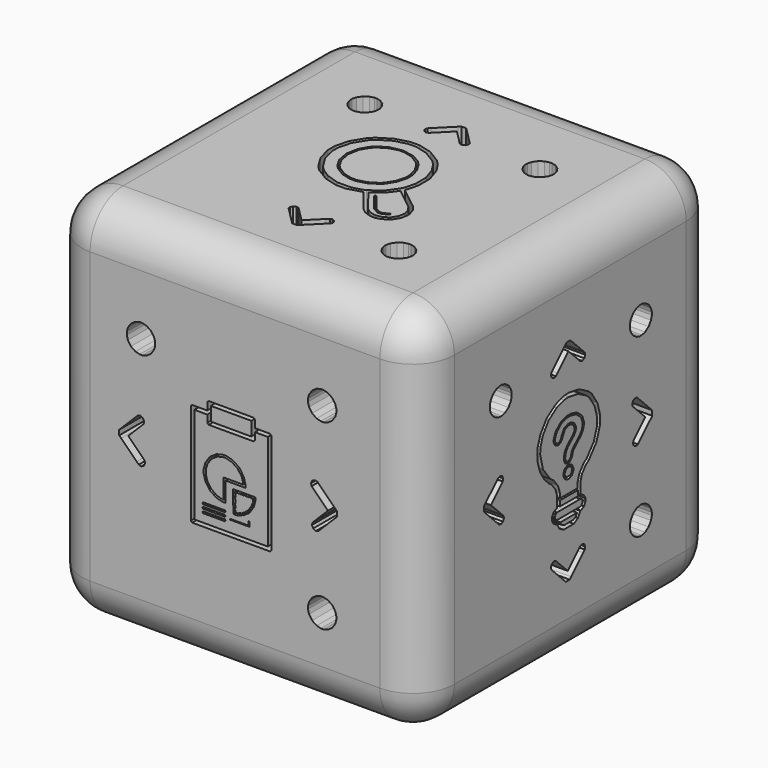
from build123d import *

# Parameters (mm, degrees)
F0_W      = 27
F0_H      = 27
F1_DEPTH  = 27
F2_R      = 3
F4_DEPTH  = 3
F5_W      = 0.6691273003
F5_H      = 0.2739462376
F5_W_2    = 0.3682261119
F5_H_2    = 4.4981792354
F5_H_3    = 0.9818197184
F6_DEPTH  = 3
F8_DEPTH  = 3
F9_W      = 1.5629880116
F9_H      = 0.1348085957
F9_W_2    = 0.0668105242
F9_H_2    = 0.385381049
F10_DEPTH = 3
F12_DEPTH = 3
F13_W     = 0.0114458475
F13_H     = 0.2253124572
F14_DEPTH = 3


# Not quite as in the source:
# - ends of sketch curves that miss each other by under 0.0002 mm in the source are joined


with BuildPart() as f1:
    # F0 (on Front) → F1 (new body)
    with BuildSketch(Plane.XZ):
        with Locations((0.4999992661, 0.4464503136)):
            Rectangle(F0_W, F0_H)
    extrude(amount=F1_DEPTH)

    # F2
    f2_edges = [f1.edges().sort_by_distance(p)[0] for p in [
        (13.999999, -13.5, 13.94645),
        (0.499999, 0, 13.94645),
        (13.999999, 0, 0.44645),
        (-13.000001, 0, 0.44645),
        (0.499999, 0, -13.05355),
        (-13.000001, -13.5, -13.05355),
        (-13.000001, -13.5, 13.94645),
        (-13.000001, -27, 0.44645),
        (13.999999, -27, 0.44645),
        (0.499999, -27, -13.05355),
        (13.999999, -13.5, -13.05355),
        (0.499999, -27, 13.94645),
    ]]
    fillet(f2_edges, radius=F2_R)

    # F3 (on face) → F4 (cut)
    with BuildSketch(Plane.XZ.offset(27)):
        Polygon((2.8811722861, -3.665039318), (-2.4466775432, -3.665039318), (-2.4466775432, 3.3292723999), (-1.5060177025, 3.3292723999), (-1.5060177025, 3.5860414556), (-2.5750279414, 3.5860414556), (-2.6071326058, 3.5860414556), (-2.7034238458, 3.4897502156), (-2.7034238458, 3.4576455512), (-2.7034238458, -3.7934352224), (-2.7034238458, -3.8255171337), (-2.6071326058, -3.9218083737), (-2.5750279414, -3.9218083737), (3.0095681906, -3.9218083737), (3.0416273487, -3.9218083737), (3.1379185887, -3.8255171337), (3.1379185887, -3.7934352224), (3.1379185887, 3.4576455512), (3.1379185887, 3.4897502156), (3.0416273487, 3.5860414556), (3.0095681906, 3.5860414556), (1.9405351985, 3.5860414556), (1.9405351985, 3.3292723999), (2.8811722861, 3.3292723999), align=None)
        Polygon((-0.2555512634, -1.8825137207), (-0.1790097389, -1.8825137207), (-0.1790097389, -0.4480882372), (1.2554157446, -0.4480882372), (1.2554157446, -0.3715467127), (1.2554157446, -0.2246752679), (1.1356887821, 0.2160073259), (0.8122303066, 0.6962348572), (0.3320482816, 1.0196478265), (-0.1086343123, 1.13814612), (-0.2555512634, 1.13814612), (-0.4024227082, 1.13814612), (-0.843105302, 1.0196478265), (-1.3233328333, 0.6962348572), (-1.6479744716, 0.2160073259), (-1.7664727651, -0.2246752679), (-1.7664727651, -0.3715467127), (-1.7664727651, -0.5184636638), (-1.6479744716, -0.9591462577), (-1.3233328333, -1.439373789), (-0.843105302, -1.7627867582), (-0.4024227082, -1.8825137207), align=None)
        Polygon((-0.3876104215, 0.98629174), (-0.2555512634, 0.98629174), (-0.1283840279, 0.98629174), (0.2555067571, 0.8875431621), (0.6789424795, 0.6135044818), (0.9739822975, 0.2061552213), (1.09370926, -0.169112128), (1.1011040267, -0.2962793635), (-0.3308186126, -0.2962793635), (-0.3308186126, -1.7282020028), (-0.4579858481, -1.7208072361), (-0.8332531974, -1.6010802736), (-1.2406024579, -1.3060404556), (-1.5146411382, -0.8826047332), (-1.6133897162, -0.4987139482), (-1.6133897162, -0.3715467127), (-1.6133897162, -0.2394875546), (-1.5072463714, 0.1567581792), (-1.2159153134, 0.5888173373), (-0.7838561553, 0.8801483953), align=None, mode=Mode.SUBTRACT)
        Polygon((7.8510243908, -6.7091576342), (7.8510243908, -6.6091576342), (7.8510243908, -6.5079517184), (7.7695454374, -6.2079744716), (7.548589806, -5.8796013203), (7.2202166547, -5.6586456889), (6.920262161, -5.5784181576), (6.820262161, -5.5784181576), (6.7190562452, -5.5784181576), (6.4190562452, -5.6586456889), (6.090705847, -5.8796013203), (5.8697502156, -6.2079744716), (5.789477178, -6.5079517184), (5.789477178, -6.6091576342), (5.789477178, -6.7091576342), (5.8697502156, -7.0091576342), (6.090705847, -7.3374852793), (6.4190562452, -7.5584409107), (6.7190562452, -7.639919864), (6.820262161, -7.639919864), (6.920262161, -7.639919864), (7.2202166547, -7.5584409107), (7.548589806, -7.3374852793), (7.7695454374, -7.0091576342), align=None)
        Polygon((7.8510243908, 6.5091813874), (7.8510243908, 6.6091586342), (7.8510243908, 6.7103873032), (7.7695454374, 7.0103417969), (7.548589806, 7.3387149482), (7.2202166547, 7.5596705796), (6.920262161, 7.6399208641), (6.820262161, 7.6399208641), (6.7190562452, 7.6399208641), (6.4190562452, 7.5596705796), (6.090705847, 7.3387149482), (5.8697502156, 7.0103417969), (5.789477178, 6.7103873032), (5.789477178, 6.6091586342), (5.789477178, 6.5091813874), (5.8697502156, 6.2092268936), (6.090705847, 5.8808537423), (6.4190562452, 5.6598981109), (6.7190562452, 5.5784191576), (6.820262161, 5.5784191576), (6.920262161, 5.5784191576), (7.2202166547, 5.6598981109), (7.548589806, 5.8808537423), (7.7695454374, 6.2092268936), align=None)
        Polygon((-5.2796923328, 6.5091813874), (-5.2796923328, 6.6091586342), (-5.2796923328, 6.7103873032), (-5.361148533, 7.0103417969), (-5.5821269175, 7.3387149482), (-5.9092486468, 7.5596705796), (-6.2092258936, 7.6399208641), (-6.3092031405, 7.6399208641), (-6.4104318094, 7.6399208641), (-6.7103863032, 7.5596705796), (-7.0387594545, 7.3387149482), (-7.2597150859, 7.0103417969), (-7.3399426172, 6.7103873032), (-7.3399426172, 6.6091586342), (-7.3399426172, 6.5091813874), (-7.2597150859, 6.2092268936), (-7.0387594545, 5.8808537423), (-6.7103863032, 5.6598981109), (-6.4104318094, 5.5784191576), (-6.3092031405, 5.5784191576), (-6.2092258936, 5.5784191576), (-5.9092486468, 5.6598981109), (-5.5821269175, 5.8808537423), (-5.361148533, 6.2092268936), align=None)
        Polygon((6.0561438447, 1.2183736513), (6.0944146069, 1.1801028891), (6.2067468026, 1.0677706934), (7.2356318993, 0.0388855967), (6.1635158584, -1.0332304443), (6.1252450961, -1.0702725375), (6.0771222292, -1.2480199778), (6.1697274625, -1.4418311268), (6.3635386115, -1.5356195228), (6.5412860518, -1.4874966559), (6.5795340609, -1.4504545626), (7.8608764954, -0.169112128), (7.8880437309, -0.1407389767), (7.8880437309, 0.2197160859), (7.8608764954, 0.2468833214), (7.747338384, 0.3592382702), (6.6227650051, 1.4837661428), (6.5104100563, 1.5961210916), (6.4721392941, 1.6343918538), (6.2943918538, 1.6825374738), (6.1005807048, 1.5899549937), (6.0080209778, 1.3961438447), align=None)
        Polygon((7.3313201815, -0.0568026854), (7.2356318993, 0.0388855967), (7.443629624, 0.2468833214), (7.443629624, -0.169112128), align=None, mode=Mode.SUBTRACT)
        Polygon((-6.0573715137, -1.0702725375), (-6.0944136069, -1.0332304443), (-6.2067458026, -0.9208754954), (-7.2356422759, 0.1080209778), (-6.1635603646, 1.1801028891), (-6.1265182713, 1.2183736513), (-6.0783498982, 1.3961438447), (-6.1709551314, 1.5899549937), (-6.3647662804, 1.6825374738), (-6.5425137207, 1.6343918538), (-6.579555814, 1.5961210916), (-7.8596695796, 0.3160073259), (-7.8880427309, 0.2888628436), (-7.8880427309, -0.071592219), (-7.8596695796, -0.1000108766), (-7.747337384, -0.2123203191), (-6.6227640051, -1.336893698), (-6.5104090563, -1.4492258936), (-6.473366963, -1.4862679869), (-6.2956195228, -1.5343908538), (-6.1018311268, -1.4430597958), (-6.0092486468, -1.2492486468), align=None)
        Polygon((-7.3313191815, 0.2036978834), (-7.2356422759, 0.1080209778), (-7.4436741303, -0.1000108766), (-7.4436741303, 0.3160073259), align=None, mode=Mode.SUBTRACT)
        Polygon((-1.5060177025, 3.5860414556), (-1.5060177025, 3.3292723999), (-1.5060177025, 2.8367354261), (-1.5060177025, 2.8058594306), (-1.4097264625, 2.7095909437), (-1.3776217981, 2.7095909437), (1.8121392941, 2.7095909437), (1.8442439585, 2.7095909437), (1.9405351985, 2.8058594306), (1.9405351985, 2.8367354261), (1.9405351985, 3.3292723999), (1.9405351985, 3.5860414556), (1.8121392941, 3.5860414556), (1.7800346297, 3.5860414556), (1.6837888959, 3.4897502156), (1.6837888959, 3.4576455512), (1.6837888959, 2.9651085774), (-1.2492486468, 2.9651085774), (-1.2492486468, 3.4576455512), (-1.2492486468, 3.4897502156), (-1.3455398868, 3.5860414556), (-1.3776217981, 3.5860414556), align=None)
        Polygon((-1.5060177025, 4.0970994761), (-1.5060177025, 3.5860414556), (-1.3776217981, 3.5860414556), (-1.3455398868, 3.5860414556), (-1.2492486468, 3.4897502156), (-1.2492486468, 3.9687035717), (1.6837888959, 3.9687035717), (1.6837888959, 3.4897502156), (1.7800346297, 3.5860414556), (1.8121392941, 3.5860414556), (1.9405351985, 3.5860414556), (1.9405351985, 4.0970994761), (1.9405351985, 4.1291813874), (1.8442439585, 4.2254726274), (1.8121392941, 4.2254726274), (-1.3776217981, 4.2254726274), (-1.4097264625, 4.2254726274), (-1.5060177025, 4.1291813874), align=None)
        Polygon((0.5245629646, -0.9764018961), (0.5246307617, -0.9702725375), (0.8418776331, -0.9702725375), (0.8418776331, -0.9542315819), (0.8455863931, -0.9517514909), (0.8480437309, -0.9480654841), (0.8850858242, -0.9480654841), (0.8887718311, -0.9517514909), (0.9069793718, -0.9702725375), (1.1578958356, -0.9702725375), (1.0850630711, -0.897439773), (1.0813543111, -0.8937310131), (1.0813543111, -0.8579403419), (1.0850630711, -0.8554602509), (1.087520409, -0.851774244), (1.1233338333, -0.851774244), (1.1270198402, -0.8554602509), (1.2418321268, -0.9702725375), (1.5331631849, -0.9702725375), (1.4924350848, -0.9295444374), (1.4887263248, -0.9258356775), (1.4887263248, -0.8900450063), (1.4924350848, -0.8875876684), (1.4948924226, -0.8838561553), (1.530705847, -0.8838561553), (1.5343918538, -0.8875876684), (1.6170826767, -0.9702725375), (1.8269743339, -0.9702725375), (1.8195340609, -1.092479591), (1.8006218933, -1.1537985395), (1.8504100563, -1.2035831177), (1.8528901473, -1.2060632088), (1.8528901473, -1.24185388), (1.8504100563, -1.2455626399), (1.8479527184, -1.2467913089), (1.8331404317, -1.2541860757), (1.8294316718, -1.2541860757), (1.8232655739, -1.2541860757), (1.8096819562, -1.2467913089), (1.8084532873, -1.2455626399), (1.7808371827, -1.2179465354), (1.712164303, -1.4406047137), (1.7985556763, -1.526996087), (1.8010585205, -1.529476178), (1.8010585205, -1.5652668493), (1.7985556763, -1.5689756092), (1.7973270074, -1.5702042782), (1.7825374738, -1.5776217981), (1.7775772918, -1.5776217981), (1.771411194, -1.5776217981), (1.7578275762, -1.5702042782), (1.7565989073, -1.5689756092), (1.6813464055, -1.4937231074), (1.5735311823, -1.6483013481), (1.6763486229, -1.7528891473), (1.6784340166, -1.7549936731), (1.8627650051, -1.481330558), (1.9825147207, -1.040625211), (1.9825147207, -0.8937310131), (1.9825147207, -0.8171894886), (0.3740278038, -0.8171894886), (0.3727991348, -0.8937310131), (0.3715477127, -1.1011030267), (0.3727991348, -1.7282020028), (0.3814453237, -2.1651985899), (0.3962348572, -2.3380313544), (0.408589806, -2.3738220256), (0.4159845728, -2.3812167924), (0.4394658015, -2.4046752679), (0.4715477127, -2.4046752679), (0.6184646638, -2.4046752679), (1.0591472577, -2.2849255523), (1.5393292827, -1.961512583), (1.6466779593, -1.8021396341), (1.6356205228, -1.7961200916), (1.6343918538, -1.7948914226), (1.5389201367, -1.6979243455), (1.4282485091, -1.8565979073), (1.415015199, -1.8656907109), (1.4887263248, -1.9393055296), (1.4912064158, -1.9417628675), (1.4912064158, -1.9775762918), (1.4887263248, -1.9812850518), (1.4862689869, -1.9825137207), (1.4714567002, -1.9911371564), (1.4677479403, -1.9911371564), (1.4615590893, -1.9911371564), (1.4479982247, -1.9825137207), (1.4467695557, -1.9812850518), (1.3652589059, -1.8998789978), (1.2086700486, -2.0074735239), (1.2751654602, -2.0750962008), (1.2776455512, -2.0775762918), (1.2776455512, -2.114595632), (1.2751654602, -2.1183043919), (1.2739367912, -2.1195330609), (1.2591245046, -2.1256991587), (1.2541870757, -2.1256991587), (1.2480209778, -2.1256991587), (1.2344373601, -2.1183043919), (1.2332086911, -2.117075723), (1.1589282278, -2.0416518666), (1.0258139243, -2.1331166786), (0.9850768939, -2.1454593946), (1.0628332645, -2.2232190677), (1.0653133555, -2.2256764056), (1.0653133555, -2.2627184989), (1.0628332645, -2.2664045057), (1.0603759266, -2.2676559278), (1.0455636399, -2.2750734477), (1.04185488, -2.2750734477), (1.0356887821, -2.2750734477), (1.0221051644, -2.2676559278), (1.0208764954, -2.2664045057), (0.9197304021, -2.1652584123), (0.7272440401, -2.2235789249), (0.7789424795, -2.2750734477), (0.7813998174, -2.2775307856), (0.7813998174, -2.3133442099), (0.7789424795, -2.3170302167), (0.7764623885, -2.3182816388), (0.7616501018, -2.3269050745), (0.7579413419, -2.3269050745), (0.7517524909, -2.3269050745), (0.7381916263, -2.3182816388), (0.7369629573, -2.3170302167), (0.6627574365, -2.2431174093), (0.6591927639, -2.2441974522), (0.5369857105, -2.2503863032), (0.5332541974, -2.2009892611), (0.5319435279, -2.1128195134), (0.4197160859, -2.0010347673), (0.4159845728, -1.9973260074), (0.4159845728, -1.961512583), (0.4197160859, -1.9590552452), (0.4221734238, -1.9553692383), (0.4579868481, -1.9553692383), (0.4616728549, -1.9590552452), (0.530679535, -2.0277897387), (0.526883258, -1.7724112682), (0.4839026615, -1.7294306718), (0.4801939016, -1.725744665), (0.4801939016, -1.6899312406), (0.4839026615, -1.6874739027), (0.4863599994, -1.6837878959), (0.5234020927, -1.6837878959), (0.5257908049, -1.6861619534), (0.5246511648, -1.3976114295), (0.4320482816, -1.3035831177), (0.4283395216, -1.2998516047), (0.4295681906, -1.2640836866), (0.4332769505, -1.2616035956), (0.4357342884, -1.2578720825), (0.4715477127, -1.2578720825), (0.4752337196, -1.2616035956), (0.5243111161, -1.311512978), (0.5234020927, -1.0813533111), (0.5236455211, -1.0593455863), (0.4715477127, -1.0073146308), (0.4678389528, -1.0035831177), (0.4678389528, -0.9678151997), (0.4715477127, -0.9653578618), (0.4740050506, -0.9616263487), (0.509818475, -0.9616263487), (0.5135044818, -0.9653578618), align=None)
        Polygon((-1.7911599096, -2.4911144033), (-0.2555512634, -2.4911144033), (-0.2394875546, -2.4911144033), (-0.1913191815, -2.4429460301), (-0.1913191815, -2.4269278276), (-0.1913191815, -2.4108641189), (-0.2394875546, -2.3626957457), (-0.2555512634, -2.3626957457), (-1.7911599096, -2.3626957457), (-1.8072236183, -2.3626957457), (-1.8541405694, -2.4108641189), (-1.8541405694, -2.4269278276), (-1.8541405694, -2.4429460301), (-1.8072236183, -2.4911144033), align=None)
        Polygon((-1.7911599096, -3.0651075774), (-0.2555512634, -3.0651075774), (-0.2394875546, -3.0651075774), (-0.1913191815, -3.0169619573), (-0.1913191815, -3.0009210017), (-0.1913191815, -2.9848800461), (-0.2394875546, -2.9367116729), (-0.2555512634, -2.9367116729), (-1.7911599096, -2.9367116729), (-1.8072236183, -2.9367116729), (-1.8541405694, -2.9848800461), (-1.8541405694, -3.0009210017), (-1.8541405694, -3.0169619573), (-1.8072236183, -3.0651075774), align=None)
        Polygon((-1.7911599096, -2.7787139482), (-0.2555512634, -2.7787139482), (-0.2394875546, -2.7787139482), (-0.1913191815, -2.7305683282), (-0.1913191815, -2.7145273726), (-0.1913191815, -2.6984636638), (-0.2394875546, -2.6503407969), (-0.2555512634, -2.6503407969), (-1.7911599096, -2.6503407969), (-1.8072236183, -2.6503407969), (-1.8541405694, -2.6984636638), (-1.8541405694, -2.7145273726), (-1.8541405694, -2.7305683282), (-1.8072236183, -2.7787139482), align=None)
        Polygon((0.1629470301, -2.8416946081), (1.5442894647, -2.8416946081), (1.5442894647, -2.5133214568), (1.5442894647, -2.50592669), (1.522036905, -2.4836741303), (1.5146421382, -2.4836741303), (1.5072473714, -2.4836741303), (1.485040318, -2.50592669), (1.485040318, -2.5133214568), (1.485040318, -2.7824454613), (0.1629470301, -2.7824454613), (0.1555295102, -2.7824454613), (0.1333224568, -2.8034238458), (0.1333224568, -2.8108186126), (0.1333224568, -2.8182133794), (0.1555295102, -2.8416946081), align=None)
        Polygon((-7.4436741303, -0.1000108766), (-7.2356422759, 0.1080209778), (-7.3313191815, 0.2036978834), (-7.4436741303, 0.3160073259), align=None)
        Polygon((7.443629624, 0.2468833214), (7.2356318993, 0.0388855967), (7.3313201815, -0.0568026854), (7.443629624, -0.169112128), align=None)
    extrude(amount=-F4_DEPTH, mode=Mode.SUBTRACT)

    # F5 (on face) → F6 (cut)
    with BuildSketch(Plane(origin=(-13.0000007339, 0, 0), x_dir=(0, -1, 0), z_dir=(-1, 0, 0))):
        Polygon((16.1785452385, -2.0737682934), (16.1121446276, -2.0737682934), (15.8333519947, -2.0737682934), (15.8333519947, 2.424410942), (16.3068997679, 2.424410942), (16.3191156816, 2.424410942), (16.3560881813, 2.4344284909), (16.3964831354, 2.4616832187), (16.4237128818, 2.5019282843), (16.4337554121, 2.5389507468), (16.4337554121, 2.5512665863), (16.4337554121, 3.1733788565), (16.4337554121, 3.1858196031), (16.4237128818, 3.2228420656), (16.3964831354, 3.2630871311), (16.3560881813, 3.2903168775), (16.3191156816, 3.3002095194), (16.3068997679, 3.3002095194), (15.8333519947, 3.3002095194), (15.8333519947, 4.4088599006), (15.8333519947, 4.4213506099), (15.8233344458, 4.458348091), (15.7960547365, 4.4985931566), (15.7556847639, 4.5258728658), (15.7186872828, 4.5357655076), (15.7063714434, 4.5357655076), (15.0842591731, 4.5357655076), (15.0719183522, 4.5357655076), (15.0349208711, 4.5258728658), (14.9945508985, 4.4985931566), (14.9672961706, 4.458348091), (14.9574035288, 4.4213506099), (14.9574035288, 4.4088599006), (14.9574035288, 3.3002095194), (13.213375744, 3.3002095194), (13.213375744, 3.574155757), (13.2467009566, 3.574155757), (13.2833237164, 3.574155757), (13.3934667915, 3.6039585895), (13.5135524713, 3.6849983118), (13.594617175, 3.8050839916), (13.624444989, 3.9152770296), (13.624444989, 3.9519997151), (13.624444989, 3.9883226979), (13.624444989, 4.0251952719), (13.594617175, 4.1353883099), (13.5135524713, 4.2554739896), (13.3934667915, 4.3364887305), (13.2833237164, 4.3661916374), (13.2467009566, 4.3661916374), (12.0033257843, 4.3661916374), (11.9665781173, 4.3661916374), (11.8564350422, 4.3364887305), (11.7363493624, 4.2554739896), (11.6552846587, 4.1353883099), (11.6255817519, 4.0251952719), (11.6255817519, 3.9883226979), (11.6255817519, 3.9519997151), (11.6255817519, 3.9152770296), (11.6552846587, 3.8050839916), (11.7363493624, 3.6849983118), (11.8564350422, 3.6039585895), (11.9665781173, 3.574155757), (12.0033257843, 3.574155757), (12.0366759782, 3.574155757), (12.0366759782, 3.3002095194), (10.057198322, 3.3002095194), (10.0447575755, 3.3002095194), (10.007735113, 3.2903168775), (9.9673401589, 3.2630871311), (9.9401104125, 3.2228420656), (9.9302177707, 3.1858196031), (9.9302177707, 3.1733788565), (9.9302177707, 2.5512665863), (9.9302177707, 2.5389507468), (9.9401104125, 2.5019282843), (9.9673401589, 2.4616832187), (10.007735113, 2.4344284909), (10.0447575755, 2.424410942), (10.057198322, 2.424410942), (12.0202631861, 2.424410942), (12.0119943366, 2.3929843173), (11.9359758794, 2.2495659924), (11.8179136946, 2.1319284917), (11.7886354718, 2.1133672976), (11.6975532192, 2.0559100345), (11.4476391063, 1.8462409873), (11.2137131015, 1.5422171215), (11.0853585721, 1.1989224655), (11.0548562599, 0.9095626925), (11.0614013916, 0.8141586544), (11.0660978983, 0.743136481), (11.1071923321, 0.5314439388), (11.2016720577, 0.26769012), (11.3398942474, 0.0277935561), (11.516887599, -0.1830995807), (11.7276558287, -0.3602428208), (11.9674274856, -0.498489992), (12.2310064344, -0.5932445132), (12.4427239581, -0.6342889841), (12.51389602, -0.6393102493), (12.5232140892, -0.6398348591), (12.6006315058, -0.643232332), (12.6265122555, -0.643232332), (12.6998327195, -0.643232332), (12.9202187954, -0.6158526971), (13.1998108337, -0.5352376589), (13.4596425697, -0.403210861), (13.6403081899, -0.2721583384), (13.6942180915, -0.2218457611), (13.7526496298, -0.1672363798), (13.9055359124, 0.0210235916), (14.061944575, 0.2998162245), (14.1589724053, 0.6041898301), (14.1923225992, 0.8442362826), (14.1923225992, 0.9242018039), (14.1923225992, 0.9826083608), (14.173336721, 1.1578530131), (14.1207508346, 1.3631752935), (14.0406604062, 1.5424919171), (13.9394107162, 1.6979762672), (13.823122212, 1.8315768945), (13.6980402485, 1.9454172196), (13.5703602175, 2.0418205144), (13.4779289682, 2.1033247673), (13.4465023435, 2.1227353296), (13.4193475413, 2.139522843), (13.3090545777, 2.2517643573), (13.2371080918, 2.3931092244), (13.2292139635, 2.424410942), (14.9574035288, 2.424410942), (14.9574035288, -2.0737682934), (10.2518535367, -2.0737682934), (10.1853030372, -2.0737682934), (9.985901353, -2.1275782693), (9.7685380288, -2.2742441786), (9.6218721195, -2.4916324842), (9.5680621436, -2.6909842056), (9.5680621436, -2.7575347051), (9.5680621436, -2.8383495946), (9.5680621436, -2.9047502056), (9.6218721195, -3.1041269083), (9.7685380288, -3.3214902326), (9.985901353, -3.4681561419), (10.1853030372, -3.5221160063), (10.2518535367, -3.5221160063), (16.1121446276, -3.5221160063), (16.1785452385, -3.5221160063), (16.3780718298, -3.4681561419), (16.5954601355, -3.3214902326), (16.7421010633, -3.1041269083), (16.7960359463, -2.9047502056), (16.7960359463, -2.8383495946), (16.7960359463, -2.7575347051), (16.7960359463, -2.6909842056), (16.7421010633, -2.4916324842), (16.5954601355, -2.2742441786), (16.3780718298, -2.1275782693), align=None)
        Polygon((16.5421747693, -2.7575347051), (16.5421747693, -2.8383495946), (16.5421747693, -2.8598835775), (16.5333563285, -2.9248102848), (16.5082999656, -3.0055752115), (16.4685795098, -3.0786208798), (16.4160186048, -3.142173609), (16.3524658756, -3.1947844768), (16.2793952259, -3.2345049326), (16.1986053177, -3.2595612956), (16.1337035919, -3.2683797364), (16.1121446276, -3.2683797364), (10.2518535367, -3.2683797364), (10.2301696652, -3.2683797364), (10.1652179766, -3.2595612956), (10.0844530499, -3.2345049326), (10.01155727, -3.1947844768), (9.9478546523, -3.142173609), (9.8952437845, -3.0786208798), (9.8555483102, -3.0055752115), (9.8304669658, -2.9248102848), (9.8217984135, -2.8598835775), (9.8217984135, -2.8383495946), (9.8217984135, -2.7575347051), (9.8217984135, -2.7358508336), (9.8304669658, -2.6709241264), (9.8555483102, -2.5901591997), (9.8952437845, -2.5172634198), (9.9478546523, -2.4535608021), (10.01155727, -2.4009499343), (10.0844530499, -2.3612794414), (10.1652179766, -2.3361731156), (10.2301696652, -2.3275045633), (10.2518535367, -2.3275045633), (15.0842591731, -2.3275045633), (15.7063714434, -2.3275045633), (16.1121446276, -2.3275045633), (16.1337035919, -2.3275045633), (16.1986053177, -2.3361731156), (16.2793952259, -2.3612794414), (16.3524658756, -2.4009499343), (16.4160186048, -2.4535608021), (16.4685795098, -2.5172634198), (16.5082999656, -2.5901591997), (16.5333563285, -2.6709241264), (16.5421747693, -2.7358508336), align=None, mode=Mode.SUBTRACT)
        Polygon((13.5699355334, 0.0095071576), (13.5210219155, -0.0363337458), (13.4716836135, -0.0823994819), (13.3047327923, -0.2004366853), (13.0637120645, -0.3147016945), (12.8039053098, -0.3773301112), (12.5990077135, -0.390620226), (12.5313830131, -0.386148552), (12.4717273852, -0.3819516737), (12.294459238, -0.3475272787), (12.0736484779, -0.2682112743), (11.8727978715, -0.1523474543), (11.6962042226, -0.0039328457), (11.5479395025, 0.1728106917), (11.4322005896, 0.3736862796), (11.3530594551, 0.5947218724), (11.3187599672, 0.7719900196), (11.3146630145, 0.831495759), (11.3119650213, 0.8698422367), (11.318210376, 1.0507826525), (11.350486369, 1.2192573403), (11.3608786391, 1.2512585377), (13.8917211878, 1.2512585377), (13.8995653533, 1.2261771933), (13.9269449882, 1.094425191), (13.9385863293, 0.9667451599), (13.9385863293, 0.9242018039), (13.9385863293, 0.8572516017), (13.9105571775, 0.6559763111), (13.8292176782, 0.400916026), (13.698190137, 0.1672398354), align=None, mode=Mode.SUBTRACT)
        Polygon((13.2795015594, 1.9275555052), (13.313251456, 1.9066710391), (13.3593421736, 1.8783670917), (13.4921433955, 1.7842870688), (13.6389591933, 1.6567569263), (13.7549479204, 1.5220321352), (13.8232721006, 1.4157861614), (13.8415335176, 1.3781141819), (11.412415306, 1.3781141819), (11.4307017045, 1.4150866816), (11.4983264049, 1.5198837332), (11.6117670273, 1.6532345463), (11.7534116714, 1.7791159152), (11.8801174272, 1.8711724431), (11.9241846498, 1.8989767622), (11.9592585616, 1.9211852434), (12.055511968, 2.0022249657), (12.1602590566, 2.1272070036), (12.235752904, 2.269351276), (12.272925255, 2.3849652819), (12.2796952195, 2.424410942), (12.9702066142, 2.424410942), (12.9767267645, 2.3849652819), (13.0131746544, 2.2692013875), (13.0866450069, 2.1277316133), (13.1876199013, 2.0050728475), align=None, mode=Mode.SUBTRACT)
        Polygon((10.1840539663, 2.6781472119), (10.1840539663, 3.0463733238), (12.1635316225, 3.0463733238), (13.0865200998, 3.0463733238), (15.0842591731, 3.0463733238), (15.7063714434, 3.0463733238), (16.1799192165, 3.0463733238), (16.1799192165, 2.6781472119), (15.7063714434, 2.6781472119), (15.0842591731, 2.6781472119), (13.0865200998, 2.6781472119), (12.1635316225, 2.6781472119), align=None, mode=Mode.SUBTRACT)
        with Locations((12.625075824, 3.4371826382)):
            Rectangle(F5_W, F5_H, mode=Mode.SUBTRACT)
        Polygon((11.8793180218, 3.9399586713), (11.8793180218, 3.9519997151), (11.8793180218, 3.9883226979), (11.8793180218, 4.0005386116), (11.8890857565, 4.0367117059), (11.9156410046, 4.076032459), (11.9550616833, 4.1027126142), (11.991259759, 4.1123554418), (12.0033257843, 4.1123554418), (13.2467009566, 4.1123554418), (13.2586420747, 4.1123554418), (13.2948401505, 4.1027126142), (13.3342608292, 4.076032459), (13.3608160773, 4.0367117059), (13.3707087191, 4.0005386116), (13.3707087191, 3.9883226979), (13.3707087191, 3.9519997151), (13.3707087191, 3.9399586713), (13.3608160773, 3.9037605955), (13.3342608292, 3.8644398425), (13.2948401505, 3.8377347059), (13.2586420747, 3.8279919526), (13.2467009566, 3.8279919526), (13.0865200998, 3.8279919526), (12.1635316225, 3.8279919526), (12.0033257843, 3.8279919526), (11.991259759, 3.8279919526), (11.9550616833, 3.8377347059), (11.9156410046, 3.8644398425), (11.8890857565, 3.9037605955), align=None, mode=Mode.SUBTRACT)
        with Locations((15.3953777618, 0.1753213243)):
            Rectangle(F5_W_2, F5_H_2, mode=Mode.SUBTRACT)
        with Locations((15.3953777618, 3.7911193785)):
            Rectangle(F5_W_2, F5_H_3, mode=Mode.SUBTRACT)
        Polygon((13.4189728201, -1.8036691942), (13.4189728201, -1.7913533548), (13.4189728201, -1.2856794772), (13.4189728201, -1.2731887678), (13.4089552711, -1.2361912867), (13.3817005433, -1.1959462211), (13.3412806078, -1.1686914933), (13.3043081081, -1.1587988515), (13.2921171758, -1.1587988515), (13.2796264665, -1.1587988515), (13.2426539668, -1.1686914933), (13.2022590127, -1.1959462211), (13.1750292663, -1.2361912867), (13.1651116431, -1.2731887678), (13.1651116431, -1.2856794772), (13.1651116431, -1.7913533548), (13.1651116431, -1.8036691942), (13.1750292663, -1.8406916568), (13.2022590127, -1.8810616294), (13.2426539668, -1.9083163572), (13.2796264665, -1.9183339061), (13.2921171758, -1.9183339061), (13.3043081081, -1.9183339061), (13.3412806078, -1.9083163572), (13.3817005433, -1.8810616294), (13.4089552711, -1.8406916568), align=None)
        Polygon((12.7518690147, -1.8036691942), (12.7518690147, -1.7913533548), (12.7518690147, -1.2856794772), (12.7518690147, -1.2731887678), (12.7418514658, -1.2361912867), (12.7145967379, -1.1959462211), (12.6743516724, -1.1686914933), (12.6373292099, -1.1587988515), (12.6250133704, -1.1587988515), (12.6125726239, -1.1587988515), (12.5755501614, -1.1686914933), (12.5353050958, -1.1959462211), (12.508050368, -1.2361912867), (12.4981577262, -1.2731887678), (12.4981577262, -1.2856794772), (12.4981577262, -1.7913533548), (12.4981577262, -1.8036691942), (12.508050368, -1.8406916568), (12.5353050958, -1.8810616294), (12.5755501614, -1.9083163572), (12.6125726239, -1.9183339061), (12.6250133704, -1.9183339061), (12.6373292099, -1.9183339061), (12.6743516724, -1.9083163572), (12.7145967379, -1.8810616294), (12.7418514658, -1.8406916568), align=None)
        Polygon((12.0849400792, -1.8036691942), (12.0849400792, -1.7913533548), (12.0849400792, -1.2856794772), (12.0849400792, -1.2731887678), (12.0748725675, -1.2361912867), (12.0476428211, -1.1959462211), (12.0073977555, -1.1686914933), (11.9704002744, -1.1587988515), (11.9580594535, -1.1587988515), (11.9455937256, -1.1587988515), (11.9085962445, -1.1686914933), (11.868176309, -1.1959462211), (11.8409465626, -1.2361912867), (11.8310539208, -1.2731887678), (11.8310539208, -1.2856794772), (11.8310539208, -1.7913533548), (11.8310539208, -1.8036691942), (11.8409465626, -1.8406916568), (11.868176309, -1.8810616294), (11.9085962445, -1.9083163572), (11.9455937256, -1.9183339061), (11.9580594535, -1.9183339061), (11.9704002744, -1.9183339061), (12.0073977555, -1.9083163572), (12.0476428211, -1.8810616294), (12.0748725675, -1.8406916568), align=None)
        Polygon((11.9171398897, 6.3705757681), (11.9388237611, 6.3921597138), (12.0322043043, 6.4855152756), (12.9660097359, 7.4191958001), (13.0593902791, 7.5126013247), (13.1471000402, 7.4248915635), (14.0243975026, 6.5477439896), (14.1122071894, 6.4599093214), (14.1337661538, 6.4383753385), (14.2161548727, 6.39103555), (14.3241995086, 6.3755970332), (14.4266732882, 6.4040508691), (14.5140582909, 6.4666792859), (14.5768365961, 6.5541142514), (14.605290432, 6.656712938), (14.5898519153, 6.7647325926), (14.5425620896, 6.8471213115), (14.5209781439, 6.8686802758), (14.4162310552, 6.9734273645), (13.3685603171, 8.0209731955), (13.263788247, 8.1257202842), (13.2441528519, 8.1454056421), (13.1689088187, 8.1879240168), (13.0595151862, 8.2086835758), (12.9500216279, 8.1880739053), (12.8746526877, 8.1454056421), (12.8550172925, 8.1257202842), (12.744549459, 8.0154273206), (11.6405206402, 6.911348539), (11.5301777138, 6.8009056869), (11.5084938423, 6.7793717039), (11.4612040167, 6.6969580036), (11.4457654999, 6.5889133676), (11.4742193359, 6.486314681), (11.5368477526, 6.3989296783), (11.6242327552, 6.3361513731), (11.7267065348, 6.3078474257), (11.8347511708, 6.3232859424), align=None)
        Polygon((6.7792364838, 5.8143644803), (6.8302985037, 5.8143644803), (6.8812605978, 5.8143644803), (7.0341468804, 5.8349741508), (7.224030644, 5.8939053175), (7.3958778234, 5.987185935), (7.5455415029, 6.1107690134), (7.6691245813, 6.2604077115), (7.7623802174, 6.4322548909), (7.8213363655, 6.6221136731), (7.8419210546, 6.7750249371), (7.8419210546, 6.8259620498), (7.8419210546, 6.8770740325), (7.8213363655, 7.0299353336), (7.7623802174, 7.2198440787), (7.6691245813, 7.3916912581), (7.5455415029, 7.5414798447), (7.3958778234, 7.6650629231), (7.224030644, 7.7583185591), (7.0341468804, 7.8172747073), (6.8812605978, 7.8377344892), (6.8302985037, 7.8377344892), (6.7792364838, 7.8377344892), (6.6263252198, 7.8172747073), (6.4364414562, 7.7583185591), (6.2645942768, 7.6650629231), (6.1148306716, 7.5414798447), (5.9913475189, 7.3916912581), (5.8981168643, 7.2198440787), (5.8391607161, 7.0299353336), (5.8187009342, 6.8770740325), (5.8187009342, 6.8259620498), (5.8187009342, 6.7750249371), (5.8391607161, 6.6221136731), (5.8981168643, 6.4322548909), (5.9913475189, 6.2604077115), (6.1148306716, 6.1107690134), (6.2645942768, 5.987185935), (6.4364414562, 5.8939053175), (6.6263252198, 5.8349741508), align=None)
        Polygon((19.6705478723, 5.8143644803), (19.721659855, 5.8143644803), (19.7726219492, 5.8143644803), (19.9254832503, 5.8349741508), (20.1153919954, 5.8939053175), (20.2872391747, 5.987185935), (20.4369777985, 6.1107690134), (20.5606108397, 6.2604077115), (20.6538414944, 6.4322548909), (20.712822624, 6.6221136731), (20.733407313, 6.7750249371), (20.733407313, 6.8259620498), (20.733407313, 6.8770740325), (20.712822624, 7.0299353336), (20.6538414944, 7.2198440787), (20.5606108397, 7.3916912581), (20.4369777985, 7.5414798447), (20.2872391747, 7.6650629231), (20.1153919954, 7.7583185591), (19.9254832503, 7.8172747073), (19.7726219492, 7.8377344892), (19.721659855, 7.8377344892), (19.6705478723, 7.8377344892), (19.5176615897, 7.8172747073), (19.3278028075, 7.7583185591), (19.1559306467, 7.6650629231), (19.0063169301, 7.5414798447), (18.8826838888, 7.3916912581), (18.7894532342, 7.2198440787), (18.7305220674, 7.0299353336), (18.7100373041, 6.8770740325), (18.7100373041, 6.8259620498), (18.7100373041, 6.7750249371), (18.7305220674, 6.6221136731), (18.7894532342, 6.4322548909), (18.8826838888, 6.2604077115), (19.0063169301, 6.1107690134), (19.1559306467, 5.987185935), (19.3278028075, 5.8939053175), (19.5176615897, 5.8349741508), align=None)
        Polygon((19.7726219492, -5.140487255), (19.721659855, -5.140487255), (19.6705478723, -5.140487255), (19.5176615897, -5.1609470369), (19.3278028075, -5.219903185), (19.1559306467, -5.3131588211), (19.0063169301, -5.4367668809), (18.8826838888, -5.586405579), (18.7894532342, -5.7582527584), (18.7305220674, -5.9481115406), (18.7100373041, -6.1010228046), (18.7100373041, -6.1520848244), (18.7100373041, -6.2030719), (18.7305220674, -6.3559332012), (18.7894532342, -6.5458169648), (18.8826838888, -6.7176891256), (19.0063169301, -6.8674527308), (19.1559306467, -6.9909109021), (19.3278028075, -7.0841665381), (19.5176615897, -7.1431226863), (19.6705478723, -7.1637323568), (19.721659855, -7.1637323568), (19.7726219492, -7.1637323568), (19.9254832503, -7.1431226863), (20.1153919954, -7.0841665381), (20.2872391747, -6.9909109021), (20.4369777985, -6.8674527308), (20.5606108397, -6.7176891256), (20.6538414944, -6.5458169648), (20.712822624, -6.3559332012), (20.733407313, -6.2030719), (20.733407313, -6.1520848244), (20.733407313, -6.1010228046), (20.712822624, -5.9481115406), (20.6538414944, -5.7582527584), (20.5606108397, -5.586405579), (20.4369777985, -5.4367668809), (20.2872391747, -5.3131588211), (20.1153919954, -5.219903185), (19.9254832503, -5.1609470369), align=None)
        Polygon((14.5953977902, -7.64784727), (13.3383328004, -6.3906323918), (13.3186724239, -6.3709969966), (13.2433034836, -6.3284286591), (13.1339348325, -6.307719063), (13.0244412743, -6.3284286591), (12.949072334, -6.3709969966), (12.929561846, -6.3906323918), (12.8191189938, -6.5009753182), (11.7148903238, -7.6051540255), (11.6045973601, -7.7156143646), (11.5829134887, -7.7371633364), (11.5356236631, -7.8195670442), (11.5201351835, -7.9275891968), (11.5486389822, -8.0300504857), (11.6113673246, -8.1174679642), (11.6986524016, -8.180221288), (11.8012510883, -8.2086826184), (11.9092707428, -8.1932316109), (11.9916594617, -8.1459292945), (12.0133683146, -8.1243828209), (12.1067238763, -8.0309972815), (13.0404293823, -7.0971818573), (13.1338099254, -7.0038013141), (13.2214947051, -7.0914860938), (14.098817149, -7.9687910507), (14.1866268358, -8.0566132282), (14.2081858001, -8.0781646981), (14.2905745191, -8.1253296167), (14.3985941736, -8.1407806241), (14.5010429717, -8.1124541935), (14.5884779372, -8.0497033678), (14.6512312611, -7.9622858893), (14.6797100784, -7.8598221023), (14.6642215988, -7.7518024478), (14.6169317732, -7.6694062344), align=None)
        Polygon((11.9916594617, -6.5535612046), (12.0133683146, -6.5320272217), (12.1067238763, -6.4386216971), (13.0404293823, -5.5047912841), (13.1338099254, -5.4114357223), (13.2214947051, -5.4990955206), (14.098817149, -6.3763929831), (14.1866268358, -6.4642276513), (14.2081858001, -6.4858115971), (14.2905745191, -6.5329515342), (14.3985941736, -6.5483900509), (14.5010429717, -6.5200861035), (14.5884779372, -6.4573077983), (14.6512312611, -6.3699227956), (14.6797100784, -6.2674490161), (14.6642215988, -6.1594043801), (14.6169317732, -6.0770156612), (14.5953977902, -6.0554566968), (14.4906007387, -5.9507096082), (13.442954982, -4.9030138886), (13.3382078933, -4.7982668), (13.3185225354, -4.7786064234), (13.2433034836, -4.7360630674), (13.1339348325, -4.7153035084), (13.0244412743, -4.7360630674), (12.949072334, -4.7786064234), (12.9294119575, -4.7982668), (12.8189691053, -4.9086097264), (11.7148903238, -6.0127884337), (11.6045973601, -6.1232312858), (11.5829134887, -6.1447652687), (11.5356236631, -6.2271789691), (11.5201351835, -6.335223605), (11.5486389822, -6.4378222917), (11.6112174361, -6.5252072944), (11.6986524016, -6.5878357111), (11.8011261812, -6.616289547), (11.9092707428, -6.6008510302), align=None)
        Polygon((6.2110590965, 0.4999673512), (6.1915486085, 0.5195028207), (6.081080775, 0.6299456728), (4.9768995696, 1.7341493615), (4.8665741301, 1.8444673065), (4.8448902586, 1.866151178), (4.7624840527, 1.9133410779), (4.6544643982, 1.9287795947), (4.5520031093, 1.9004506659), (4.4645806345, 1.8376973421), (4.4018298089, 1.7502623766), (4.3733684785, 1.647788597), (4.388819486, 1.5397939239), (4.4361193042, 1.4573802235), (4.4578056738, 1.4356963521), (4.5511887151, 1.3423407903), (5.4850091355, 0.4085103773), (5.5784046676, 0.3151048527), (5.4905650031, 0.227420073), (4.613397444, -0.6497275009), (4.525707668, -0.7375871505), (4.5040212984, -0.7591211335), (4.4567239784, -0.8415348338), (4.4412729709, -0.9495295069), (4.4697343012, -1.0521281936), (4.5323502272, -1.1395631591), (4.6197677057, -1.2021665944), (4.7222314928, -1.2306454117), (4.8303860469, -1.2151819135), (4.9127897547, -1.1678920879), (4.9344761243, -1.1463331236), (5.0391058003, -1.0415610535), (6.0867765384, 0.0059597961), (6.1915486085, 0.1107568476), (6.2110590965, 0.1303922428), (6.253627434, 0.2057362016), (6.2743620116, 0.3151048527), (6.253627434, 0.4246233924), align=None)
        Polygon((6.5692926409, 1.7341493615), (6.4589497145, 1.8444673065), (6.437265843, 1.866151178), (6.3548521427, 1.913465985), (6.2468324881, 1.9289045018), (6.14438369, 1.9004506659), (6.0569487245, 1.8376973421), (5.9942203821, 1.7503872836), (5.9657415647, 1.647788597), (5.9812050629, 1.5397939239), (6.0284948886, 1.4573802235), (6.05017876, 1.4356963521), (6.1435593032, 1.3423407903), (7.0773647348, 0.4085103773), (7.1707702593, 0.3151048527), (7.0829355911, 0.227420073), (6.2056381287, -0.6497275009), (6.117953349, -0.7375871505), (6.0962694775, -0.7591211335), (6.049104559, -0.8415348338), (6.0336410608, -0.9495295069), (6.0619699896, -1.0520032865), (6.1247233135, -1.139438252), (6.2121332975, -1.2021665944), (6.3146070771, -1.2306454117), (6.4227516387, -1.2151819135), (6.5051653391, -1.1678920879), (6.5268492105, -1.1463331236), (6.6314963735, -1.0415610535), (7.6791421302, 0.0061096846), (7.7839391817, 0.1107568476), (7.8034246883, 0.1303922428), (7.8459930258, 0.2057362016), (7.8667276033, 0.3151048527), (7.8459930258, 0.4246233924), (7.8034246883, 0.4999673512), (7.7839391817, 0.5195028207), (7.6734713482, 0.6299456728), align=None)
        Polygon((22.3601972998, -0.7591211335), (22.3386633168, -0.7375871505), (22.2452577922, -0.6441816259), (21.3114273792, 0.2896487871), (21.2180718175, 0.3828794417), (21.3057565972, 0.4707141099), (22.1830790411, 1.3480115724), (22.2708887278, 1.4356963521), (22.2924476922, 1.4573802235), (22.3395876293, 1.5397939239), (22.3550761089, 1.647788597), (22.3267221987, 1.7502623766), (22.2639938563, 1.8376973421), (22.1765588908, 1.9004506659), (22.0741100926, 1.9289045018), (21.9660904381, 1.913465985), (21.8836767378, 1.866151178), (21.8621427548, 1.8444673065), (21.7573706847, 1.7397202179), (20.7096999466, 0.6921494054), (20.6049278765, 0.5874023167), (20.5852675, 0.5678668473), (20.5426991625, 0.4925228885), (20.5219895664, 0.3831542373), (20.5426991625, 0.2736356977), (20.5852675, 0.1982917388), (20.6049278765, 0.1786563437), (20.7152458216, 0.0683134172), (21.8194245288, -1.03586529), (21.9298923624, -1.1463331236), (21.9514513267, -1.1678920879), (22.0338650271, -1.2151819135), (22.1418597002, -1.2306454117), (22.2444583868, -1.2021665944), (22.3318933524, -1.1395631591), (22.3944967877, -1.0521281936), (22.422975605, -0.9495295069), (22.4075121068, -0.8415348338), align=None)
        Polygon((19.7190867689, 0.2894988986), (19.6256812443, 0.3828794417), (19.7133910054, 0.4707141099), (20.5906884679, 1.3480115724), (20.6784981546, 1.4356963521), (20.700057119, 1.4573802235), (20.7472470189, 1.5397939239), (20.7626855357, 1.647788597), (20.7343566069, 1.7502623766), (20.6716032831, 1.8376973421), (20.5841683176, 1.9004506659), (20.4817195194, 1.9289045018), (20.3736998649, 1.913465985), (20.2912861645, 1.866151178), (20.2697521816, 1.8444673065), (20.1649551301, 1.7397202179), (19.1173093734, 0.6920244983), (19.0125622847, 0.5872774097), (18.9928769268, 0.5677419402), (18.9503585521, 0.4925228885), (18.9295989932, 0.3830043488), (18.9503585521, 0.2736356977), (18.9928769268, 0.1981418503), (19.0125622847, 0.1785064552), (19.1228552484, 0.0681885102), (20.2270839184, -1.03586529), (20.3375017892, -1.1463331236), (20.3590607535, -1.1678920879), (20.4414744539, -1.2151819135), (20.549469127, -1.2306454117), (20.651967888, -1.2021665944), (20.7395027791, -1.1395631591), (20.8021311959, -1.0521281936), (20.8305850318, -0.9496793954), (20.815146515, -0.8415348338), (20.7678067265, -0.7591211335), (20.7462727436, -0.7375871505), (20.6528922005, -0.6441816259), align=None)
    extrude(amount=-F6_DEPTH, mode=Mode.SUBTRACT)

    # F7 (on face) → F8 (cut)
    with BuildSketch(Plane(origin=(0, 0, 0), x_dir=(-1, 0, 0), z_dir=(0, 1, 0))):
        Polygon((-0.6705348159, -1.7825302972), (-0.4712687987, -1.7825302972), (-0.3316880227, -1.7825302972), (0.0882858356, -1.6942339658), (0.1384047246, -1.6775203389), (0.2541465907, -1.6369678021), (0.7552475141, -1.3136250971), (1.1322717497, -0.8495140688), (1.1859532802, -0.7397319303), (1.2384472636, -0.6288062277), (1.364943029, -0.0453467087), (1.3040922323, 0.5476351793), (1.2635177039, 0.6633550538), (1.2229431755, 0.7790969198), (0.8996004704, 1.2814073821), (0.4366769894, 1.6584096261), (0.3268948508, 1.710925601), (0.1658502593, 1.788468033), (-0.3806193645, 1.8910809054), (-1.0773796804, 1.7896775718), (-1.6858876481, 1.4341391434), (-2.0485953428, 1.0129337547), (-2.1261377748, 0.8518891632), (-2.2037021985, 0.6920101272), (-2.305105532, 0.1455405034), (-2.2025146513, -0.5512198125), (-1.8469542313, -1.1597057886), (-1.4269583814, -1.5224134832), (-1.2659137898, -1.5999779069), (-1.2038754459, -1.6298205275), align=None)
        Polygon((-0.6764945433, 1.6417179908), (-0.4677061572, 1.6417179908), (-0.3114117543, 1.6417179908), (0.1610780789, 1.5116815755), (0.2171566954, 1.4842360408), (0.3126003015, 1.4389113237), (0.7122978914, 1.1143810715), (0.9902718962, 0.6812562278), (1.0260742443, 0.5810404415), (1.0606890452, 0.4808246551), (1.1143705757, -0.032217715), (1.0046104287, -0.535737716), (0.9592857116, -0.6311813221), (0.9127294642, -0.7266249281), (0.5870116647, -1.1263225181), (0.1538868211, -1.4043185144), (0.0548805735, -1.4400988709), (-0.0453352129, -1.4747136718), (-0.5583775829, -1.5272076551), (-1.0618755923, -1.4186350553), (-1.1573191984, -1.3733103383), (-1.2527628045, -1.3267540908), (-1.6524603944, -1.0010362914), (-1.9316659296, -0.5679334393), (-1.9662807305, -0.4689052001), (-2.0020830786, -0.3686894138), (-2.0545550703, 0.1443529563), (-1.9447949233, 0.6478509657), (-1.8982606674, 0.7432945718), (-1.830262596, 0.8852944253), (-1.3029036851, 1.40548407), align=None, mode=Mode.SUBTRACT)
        Polygon((-2.9147790553, 1.6011434624), (-2.7883272731, 1.6011434624), (-2.7000309416, 1.6011434624), (-2.435163939, 1.6560345317), (-2.4029682157, 1.6667884311), (-2.3301759723, 1.693024427), (-2.0116054476, 1.8982501716), (-1.7729964324, 2.1917502561), (-1.7383816315, 2.2609578663), (-1.6894502897, 2.363548747), (-1.6250368514, 2.7095648064), (-1.6906598284, 3.1498149331), (-1.9161618415, 3.5352179738), (-2.1822163913, 3.7654921671), (-2.2836197248, 3.8131919785), (-2.3862545888, 3.8621233204), (-2.7310611094, 3.9277462974), (-3.1725207749, 3.8633328591), (-3.5579018239, 3.6378088545), (-3.7869664785, 3.3717543047), (-3.8358978203, 3.2691634239), (-3.870468638, 3.1999338221), (-3.9122527052, 2.4542421644), (-3.8859947177, 2.3802623739), (-3.860946269, 2.3074701306), (-3.6557205243, 1.9901311362), (-3.3622204399, 1.7514781378), (-3.2918252825, 1.7168853285), (-3.2524602929, 1.6977966073), align=None)
        Polygon((-2.9064442335, 3.6760082885), (-2.7859521787, 3.6760082885), (-2.6964683001, 3.6760082885), (-2.4244320312, 3.602028498), (-2.3922143163, 3.5865024183), (-2.2800570833, 3.5327988962), (-1.9281032881, 3.0663127736), (-1.9125772084, 2.484084785), (-1.9662807305, 2.3707400049), (-1.9925167263, 2.3158489356), (-2.4292042115, 1.9244861675), (-2.4864703752, 1.9042098991), (-2.5437365388, 1.8851211779), (-3.128383605, 1.9173388929), (-3.1832306911, 1.9435748887), (-3.2381217604, 1.9698548678), (-3.6282969813, 2.4064983698), (-3.6473857025, 2.4637645334), (-3.6676619709, 2.5210526886), (-3.6366318031, 3.1056777632), (-3.6092082601, 3.1605688325), (-3.5710308177, 3.2428834449), (-3.2667768338, 3.5411777012), align=None, mode=Mode.SUBTRACT)
        Polygon((7.5882619937, 6.2197343315), (7.5882619937, 6.3163654848), (7.5882619937, 6.4142061768), (7.5095100229, 6.7041436197), (7.2959494564, 7.0215046057), (6.9785664788, 7.2350651722), (6.6886510275, 7.3126076042), (6.5919978826, 7.3126076042), (6.4941791822, 7.3126076042), (6.2042197476, 7.2350651722), (5.8868587616, 7.0215046057), (5.6732981952, 6.7041436197), (5.5957117799, 6.4142061768), (5.5957117799, 6.3163654848), (5.5957117799, 6.2197343315), (5.6732981952, 5.9297968886), (5.8868587616, 5.612413911), (6.2042197476, 5.3988533445), (6.4941791822, 5.3201233653), (6.5919978826, 5.3201233653), (6.6886510275, 5.3201233653), (6.9785664788, 5.3988533445), (7.2959494564, 5.612413911), (7.5095100229, 5.9297968886), align=None)
        Polygon((7.5882619937, -6.5562060303), (7.5882619937, -6.4595748771), (7.5882619937, -6.3617341851), (7.5095100229, -6.0718187337), (7.2959494564, -5.7544357561), (6.9785664788, -5.5408751896), (6.6886510275, -5.463310766), (6.5919978826, -5.463310766), (6.4941791822, -5.463310766), (6.2042197476, -5.5408751896), (5.8868587616, -5.7544357561), (5.6732981952, -6.0718187337), (5.5957117799, -6.3617341851), (5.5957117799, -6.4595748771), (5.5957117799, -6.5562060303), (5.6732981952, -6.8461434733), (5.8868587616, -7.1635044593), (6.2042197476, -7.3770870173), (6.4941791822, -7.4558169965), (6.5919978826, -7.4558169965), (6.6886510275, -7.4558169965), (6.9785664788, -7.3770870173), (7.2959494564, -7.1635044593), (7.5095100229, -6.8461434733), align=None)
        Polygon((-5.1029886615, 6.2197343315), (-5.1029886615, 6.3163654848), (-5.1029886615, 6.4142061768), (-5.1817186407, 6.7041436197), (-5.3953011988, 7.0215046057), (-5.7114746376, 7.2350651722), (-6.0014120805, 7.3126076042), (-6.0980432338, 7.3126076042), (-6.1958839258, 7.3126076042), (-6.4857993771, 7.2350651722), (-6.8031823547, 7.0215046057), (-7.0167429212, 6.7041436197), (-7.0942853532, 6.4142061768), (-7.0942853532, 6.3163654848), (-7.0942853532, 6.2197343315), (-7.0167429212, 5.9297968886), (-6.8031823547, 5.612413911), (-6.4857993771, 5.3988533445), (-6.1958839258, 5.3201233653), (-6.0980432338, 5.3201233653), (-6.0014120805, 5.3201233653), (-5.7114746376, 5.3988533445), (-5.3953011988, 5.612413911), (-5.1817186407, 5.9297968886), align=None)
        Polygon((-0.9413835376, -3.7213769888), (-0.839980204, -3.7213769888), (-0.7170690717, -3.7213769888), (-0.3460265552, -3.5805646825), (-0.0322062191, -3.2727480571), (0.0083463176, -3.189223906), (0.0644249341, -3.0723164843), (0.0465457517, -2.4721433384), (-0.3161839346, -1.9925282221), (-0.4319038091, -1.9364496057), (-0.5488332223, -1.8803709892), (-1.1489843766, -1.8970626245), (-1.6286214845, -2.2597923108), (-1.684700101, -2.3766997324), (-1.7407787174, -2.4924415984), (-1.7240650906, -3.0925927527), (-1.3625449431, -3.5722298606), (-1.2456155298, -3.6294960243), (-1.2133978149, -3.6450001124), align=None)
        Polygon((-0.9270450051, -2.09630665), (-0.8363735793, -2.09630665), (-0.7683755079, -2.09630665), (-0.5643373104, -2.1523852665), (-0.5404984005, -2.1643267131), (-0.4557867022, -2.2049012415), (-0.1909196996, -2.5556674896), (-0.178978253, -2.9947300691), (-0.2195307898, -3.0806513062), (-0.2612928653, -3.1653410128), (-0.612081105, -3.4302300071), (-1.0511436846, -3.4421714537), (-1.1358553829, -3.4015969253), (-1.2217766199, -3.3598568413), (-1.4866436226, -3.00904661), (-1.4985630775, -2.5699840305), (-1.456801002, -2.4852943238), (-1.4281459285, -2.4232559799), (-1.199081274, -2.1977539668), align=None, mode=Mode.SUBTRACT)
        Polygon((-1.1060347539, 5.8534420037), (-1.0690448586, 5.8892443518), (-0.9604722588, 5.9978169516), (0.0329461519, 6.9923219231), (1.0702114142, 5.9560328844), (1.1060137622, 5.9202745196), (1.2778122532, 5.8737182721), (1.4651368238, 5.9632241423), (1.554642694, 6.1505487129), (1.5080864465, 6.3223472038), (1.4722840984, 6.3581275603), (0.2350578695, 7.5965853197), (0.2075903432, 7.6240528459), (-0.1408008106, 7.6240528459), (-0.1682243536, 7.5965853197), (-1.4723270817, 6.2913170361), (-1.5093169769, 6.255514688), (-1.5558292412, 6.0837161971), (-1.4663453626, 5.8963916264), (-1.2790427836, 5.8069297395), align=None)
        Polygon((0.1252757309, 7.0847524884), (0.0329461519, 6.9923219231), (-0.1682243536, 7.1933030966), (0.2350578695, 7.1933030966), align=None, mode=Mode.SUBTRACT)
        Polygon((5.8534534995, 1.1060022664), (5.8904433948, 1.0690123712), (5.9990159946, 0.960461763), (6.9935732203, -0.0340954627), (5.9572319274, -1.0714314488), (5.9202420322, -1.1072337968), (5.8737297679, -1.2790542794), (5.9632356381, -1.4663348668), (6.1505602087, -1.555840737), (6.3223586996, -1.5093284727), (6.3593266033, -1.4735261246), (7.5977843627, -0.2362559124), (7.6240423501, -0.2088103778), (7.6240423501, 0.1396027676), (7.5977843627, 0.1670263106), (7.4880462073, 0.2755989104), (6.4011106705, 1.3625344473), (6.292516079, 1.4710850555), (6.2555261838, 1.5080749507), (6.0837276929, 1.5546311982), (5.8964031222, 1.4651473196), (5.8069412353, 1.277822749), align=None)
        Polygon((7.0859515314, -0.1264737738), (6.9935732203, -0.0340954627), (7.1945021396, 0.1670263106), (7.1945021396, -0.2362559124), align=None, mode=Mode.SUBTRACT)
        Polygon((1.1060137622, -5.8546515425), (1.0702114142, -5.8916414378), (0.9604732588, -6.0002140376), (-0.0334610796, -6.9941483759), (-0.9676195334, -6.0610648343), (-1.0702324058, -5.9584739536), (-1.107222301, -5.9214840584), (-1.2790427836, -5.8749278109), (-1.4663453626, -5.9644336811), (-1.5558292412, -6.1517582517), (-1.5093169769, -6.3235567426), (-1.4723270817, -6.3605466379), (-1.3696922177, -6.4631375186), (-0.3388352973, -7.493994439), (-0.2350568695, -7.5978168501), (-0.2076113348, -7.6240528459), (0.1408018106, -7.6240528459), (0.1682253536, -7.5978168501), (0.2767979534, -7.4892442503), (1.3637334902, -6.4023087134), (1.4722840984, -6.293714122), (1.5080864465, -6.2567242268), (1.554642694, -6.0849257358), (1.4651368238, -5.8976231568), (1.2778122532, -5.8081392783), align=None)
        Polygon((-0.126462278, -7.0871495744), (-0.0334610796, -6.9941483759), (0.0644249341, -7.0919217547), (0.1682253536, -7.1957441658), (-0.2350568695, -7.1957441658), align=None, mode=Mode.SUBTRACT)
        Polygon((-5.8546400467, -1.1072337968), (-5.8904423948, -1.0714314488), (-5.9990149946, -0.9616713018), (-6.9929989434, 0.032312647), (-5.9572749106, 1.0690123712), (-5.9214725626, 1.1060022664), (-5.8749163151, 1.277822749), (-5.9644221853, 1.4651473196), (-6.1517467559, 1.5546311982), (-6.3235452468, 1.5080749507), (-6.3593475949, 1.4710850555), (-7.5966178071, 0.2338588265), (-7.6240413501, 0.2075788474), (-7.6240413501, -0.1419998535), (-7.5966178071, -0.1694233966), (-7.4880452073, -0.2779959964), (-6.4011096705, -1.363743986), (-6.292515079, -1.4735261246), (-6.256712731, -1.5093284727), (-6.08491424, -1.555840737), (-5.897611661, -1.4663348668), (-5.8081277824, -1.2790542794), align=None)
        Polygon((-7.0859505314, 0.1252642351), (-6.9929989434, 0.032312647), (-7.1945451228, -0.1694233966), (-7.1945451228, 0.2338588265), align=None, mode=Mode.SUBTRACT)
        Polygon((2.0998807874, -1.1478083252), (2.1738605779, -1.1478083252), (2.225167014, -1.1478083252), (2.3802738697, -1.1143810715), (2.3993625909, -1.108421344), (2.4423122136, -1.0929172559), (2.7680300131, -0.8017922658), (2.7883062814, -0.7612177374), (2.8073950027, -0.7194556619), (2.8312778958, -0.2839557239), (2.8169613549, -0.2422156399), (2.8014352752, -0.1992660172), (2.5103322767, 0.127661321), (2.4697577483, 0.1467500422), (2.4280176643, 0.1670263106), (1.9913301792, 0.1908872121), (1.949546112, 0.1753831241), (1.9065964893, 0.1610665831), (1.5796911427, -0.130058407), (1.5606024215, -0.1718424741), (1.5403261531, -0.2123950109), (1.5164652516, -0.6490824961), (1.5319693396, -0.6920321188), (1.5462638889, -0.7349597499), (1.8374108707, -1.0594900022), (1.8791729462, -1.0797882622), (1.901824309, -1.0905421616), align=None)
        Polygon((2.139245777, -0.038199434), (2.175048125, -0.038199434), (2.2168102006, -0.038199434), (2.3444715216, -0.0739797905), (2.3599976013, -0.0811490568), (2.38504605, -0.0930685117), (2.5687859875, -0.2982722648), (2.5783083565, -0.325739791), (2.5878747087, -0.3519757869), (2.5723706206, -0.6263871501), (2.5604291741, -0.6526451376), (2.5341931782, -0.7051611126), (2.3158604314, -0.8709778844), (2.0414270765, -0.8781691423), (1.9889330932, -0.8530767104), (1.9626751057, -0.8399697082), (1.7789571599, -0.6347439636), (1.7705783548, -0.6084859761), (1.7610559858, -0.5810624331), (1.7753505351, -0.3054635226), (1.7884795289, -0.2803930823), (1.8004209754, -0.2541570865), (2.0044371813, -0.0715827046), (2.0318827159, -0.0620603356), (2.0438021709, -0.0572881553), align=None, mode=Mode.SUBTRACT)
        Polygon((3.4325946056, -0.0298426206), (3.4922578552, -0.0298426206), (3.5638405598, -0.0298426206), (3.7821733066, 0.0524939833), (3.9671227828, 0.2338588265), (3.9909836843, 0.2827461851), (4.0064877724, 0.3161734388), (4.0255764936, 0.6693147813), (4.0136790303, 0.7039295822), (4.0017375837, 0.7385223915), (3.7655036629, 1.0034113857), (3.7320764092, 1.0189154738), (3.662868799, 1.0523427275), (3.3109150037, 1.0415888281), (3.028146827, 0.8292158088), (2.9959071204, 0.7600081986), (2.9625238499, 0.6920101272), (2.9732557577, 0.3400123487), (3.185628777, 0.057244172), (3.2548363872, 0.0238609015), (3.2739251084, 0.0155040881), align=None)
        Polygon((3.4266568698, 0.8208370038), (3.4946329496, 0.8208370038), (3.523288023, 0.8208370038), (3.6127719016, 0.7969980939), (3.6235038094, 0.7910383664), (3.6414049834, 0.7826595614), (3.7690663044, 0.6395161439), (3.7762135791, 0.6204054311), (3.7821733066, 0.6025262486), (3.7726509376, 0.4104294977), (3.7643161157, 0.3913407765), (3.7452273945, 0.3543508812), (3.5924956332, 0.2386090152), (3.4003768907, 0.2338588265), (3.363408987, 0.2517600005), (3.3455298046, 0.2600948223), (3.2166589448, 0.4032822231), (3.2106992173, 0.4223709443), (3.2035299511, 0.4414596655), (3.2142838505, 0.6335564164), (3.2238062195, 0.6514575904), (3.235747666, 0.6788811335), align=None, mode=Mode.SUBTRACT)
        Polygon((-2.7811580068, 0.4414596655), (-2.7215167488, 0.4414596655), (-2.6797546733, 0.4414596655), (-2.5532808994, 0.4676956613), (-2.5377768113, 0.4724678416), (-2.503184002, 0.4855968354), (-2.2406920937, 0.7218307562), (-2.2239784669, 0.7540484712), (-2.2084523872, 0.7874537333), (-2.1881761188, 1.1418046145), (-2.2001175653, 1.1763974238), (-2.2132465591, 1.2110122247), (-2.4494804799, 1.4746916802), (-2.4816981949, 1.4901957683), (-2.5508838134, 1.5236010304), (-2.9040691391, 1.5140786614), (-3.1856497686, 1.3017056421), (-3.217845492, 1.2324760403), (-3.2345591188, 1.2002583253), (-3.2548353872, 0.8459294357), (-3.2417063935, 0.8113146348), (-3.2297869385, 0.7766998339), (-2.9935310261, 0.5130203784), (-2.9601477556, 0.4963067515), (-2.9410590344, 0.4879719297), align=None)
        Polygon((-2.7883272731, 1.2933268371), (-2.72030721, 1.2933268371), (-2.6905085726, 1.2933268371), (-2.6010027024, 1.2694659355), (-2.590248803, 1.2635281997), (-2.5532808994, 1.2456270256), (-2.4387265805, 1.0928952643), (-2.432766853, 0.9020080522), (-2.4506680271, 0.8638306098), (-2.4602343793, 0.8459294357), (-2.6033997884, 0.7182461231), (-2.6213009624, 0.7110988484), (-2.6403896837, 0.7051171293), (-2.832464443, 0.7146834816), (-2.850365617, 0.7230183034), (-2.8694543382, 0.7325846556), (-2.998325198, 0.8757280731), (-3.0042849255, 0.8948167943), (-3.0114322001, 0.9139055155), (-3.0007002924, 1.1048147193), (-2.9911559318, 1.1227158933), (-2.9792364768, 1.150161428), align=None, mode=Mode.SUBTRACT)
        Polygon((2.2645320036, 0.7182461231), (2.2836427165, 0.7182461231), (2.287205358, 0.7182461231), (2.3003343517, 0.7206212174), (2.3027314377, 0.7206212174), (2.3122538067, 0.7230183034), (2.3599976013, 0.8029578214), (2.3576005154, 0.812502182), (2.3003343517, 1.0439639225), (1.9746165523, 1.6977966073), (1.3422696747, 2.3886411789), (0.5202011405, 2.8384136746), (-0.1932947939, 2.9982927106), (-0.4307162619, 2.9982927106), (-0.6395046481, 2.9982927106), (-1.2623291567, 2.8778006558), (-1.3351214, 2.8527522072), (-1.3458313162, 2.8503551212), (-1.3864058446, 2.7668309701), (-1.3828212115, 2.7560990623), (-1.3804461171, 2.7465547017), (-1.2981315048, 2.7059801733), (-1.2873776054, 2.7083772593), (-1.219379534, 2.731028622), (-0.6454643755, 2.8455609493), (-0.4307162619, 2.8455609493), (-0.206401796, 2.8455609493), (0.4688947043, 2.69408271), (1.2480136158, 2.268105141), (1.8469552313, 1.6142944478), (2.1559594038, 0.9950765639), (2.209662926, 0.7755122867), (2.2108504731, 0.7671774649), align=None)
        Polygon((-2.3325510667, -2.2037136943), (-2.3206096201, -2.2037136943), (-2.3075246096, -2.2037136943), (-2.2657405424, -2.1798527928), (-2.2609683621, -2.1750806125), (-2.2550086346, -2.166723799), (-2.2645310036, -2.0748428345), (-2.2729098087, -2.068883107), (-2.435163939, -1.9388247), (-3.0233736467, -1.1239254321), (-3.2882406494, -0.2422156399), (-3.2882406494, 0.0512844446), (-3.2882406494, 0.107363061), (-3.2798838359, 0.2720362689), (-3.27748675, 0.2911249901), (-3.27748675, 0.3018349063), (-3.3371499996, 0.3734396024), (-3.347903899, 0.3734396024), (-3.3586577983, 0.3746271496), (-3.4290309641, 0.3161734388), (-3.4290309641, 0.3054195394), (-3.4314060585, 0.285143271), (-3.4409724107, 0.1157198745), (-3.4409724107, 0.0512844446), (-3.4409724107, -0.2589072752), (-3.1605793283, -1.1895484092), (-2.5389863501, -2.0497943858), (-2.3683534147, -2.1870000674), (-2.3647907732, -2.1893751618), align=None)
        Polygon((0.5702980379, -2.6714313472), (0.5881992119, -2.6714313472), (0.5941589394, -2.6714313472), (0.6132476606, -2.6666371753), (0.6156667382, -2.6666371753), (0.751662881, -2.6129336532), (1.3673181234, -2.2359314092), (1.8744007659, -1.7204919532), (1.9579029254, -1.5987903597), (1.9638626529, -1.5892459991), (1.9459614789, -1.4997621205), (1.937626657, -1.493802393), (1.9280603048, -1.4878426655), (1.8374108707, -1.5045343008), (1.8314291516, -1.5140786614), (1.7526771808, -1.6286329803), (1.2730620645, -2.1165829184), (0.6896025455, -2.4745404244), (0.5607756689, -2.5246593134), (0.5500217695, -2.5282439465), (0.5130318742, -2.611746106), (0.5178040545, -2.6225000054), (0.5202011405, -2.6296472801), align=None)
        Polygon((0.0644249341, -7.0919217547), (-0.0334610796, -6.9941483759), (-0.126462278, -7.0871495744), (-0.2350568695, -7.1957441658), (0.1682253536, -7.1957441658), align=None)
        Polygon((-7.1945451228, -0.1694233966), (-6.9929989434, 0.032312647), (-7.0859505314, 0.1252642351), (-7.1945451228, 0.2338588265), align=None)
        Polygon((-0.1682243536, 7.1933030966), (0.0329461519, 6.9923219231), (0.1252757309, 7.0847524884), (0.2350578695, 7.1933030966), align=None)
        Polygon((7.1945021396, 0.1670263106), (6.9935732203, -0.0340954627), (7.0859515314, -0.1264737738), (7.1945021396, -0.2362559124), align=None)
    extrude(amount=-F8_DEPTH, mode=Mode.SUBTRACT)

    # F9 (on face) → F10 (cut)
    with BuildSketch(Plane.YZ.offset(13.9999992661)):
        Polygon((-14.561439243, -2.0796370229), (-14.4266086558, -2.0796370229), (-14.4266086558, -1.9567258905), (-14.4266086558, -1.7682137727), (-14.6151427652, -1.2038869582), (-15.0255502713, -0.687259955), (-15.136519957, -0.6084859926), (-15.3226569805, -0.4760744829), (-15.9776772124, 0.3961129403), (-16.2294152213, 1.4603751228), (-16.2115140473, 1.687064683), (-16.1948004204, 1.9137762349), (-15.9776772124, 2.5783188358), (-15.4586751149, 3.3120910386), (-14.7212962874, 3.8263429474), (-14.0555441477, 4.0399035139), (-13.8288545874, 4.055407602), (-13.6486992831, 4.0685585873), (-12.7860782121, 3.9170143732), (-12.0224853804, 3.4934338901), (-11.8900298874, 3.370566741), (-11.7599714804, 3.2500746863), (-11.2863160916, 2.5138834059), (-11.0715459864, 1.7455403855), (-11.0715459864, 1.488986213), (-11.0715459864, 1.191923487), (-11.3650460708, 0.2970847011), (-12.0033966591, -0.5047075647), (-12.1763826972, -0.6251996194), (-12.2849772887, -0.6991794099), (-12.682255801, -1.2062620525), (-12.8636206441, -1.7789676721), (-12.8636206441, -1.9698548843), (-12.8636206441, -2.0796370229), (-12.7288120485, -2.0796370229), (-12.7120984216, -2.0796370229), (-12.6607919854, -2.1297339202), (-12.6607919854, -2.1464255555), (-12.6607919854, -2.5998266675), (-12.6309713565, -2.5998266675), (-12.5939814612, -2.5998266675), (-12.5939814612, -1.9698548843), (-12.5939814612, -1.8099538567), (-12.4424592387, -1.3303387404), (-12.1119472673, -0.9079677961), (-12.0224853804, -0.8459294522), (-11.8315761766, -0.7123084037), (-11.1264370557, 0.1729860216), (-10.8019068034, 1.1608933193), (-10.8019068034, 1.488986213), (-10.8019068034, 1.7729639285), (-11.0393282714, 2.6224779973), (-11.5631245408, 3.4337926321), (-11.7062899499, 3.5674136806), (-11.851852445, 3.7034318151), (-12.6965723419, 4.171149468), (-13.6486992831, 4.3381977703), (-13.8479433087, 4.3238592377), (-14.0972842316, 4.3071676025), (-14.8334535203, 4.0709336817), (-15.6483747799, 3.5030002423), (-16.2210803995, 2.6916636159), (-16.462064509, 1.956703866), (-16.4799656831, 1.707362943), (-16.494282224, 1.5247885611), (-16.4417882406, 0.9699841155), (-16.2222679467, 0.2827461686), (-15.8344898117, -0.3269273547), (-15.4419614881, -0.7218307727), (-15.2928143599, -0.8280282781), (-15.1997458481, -0.8936512552), (-14.8549393275, -1.3267541073), (-14.6962698303, -1.7992439405), (-14.6962698303, -1.9567258905), (-14.6962698303, -2.5998266675), (-14.6592799351, -2.5998266675), (-14.6282497673, -2.5998266675), (-14.6282497673, -2.1464255555), (-14.6282497673, -2.1297339202), (-14.5781528699, -2.0796370229), align=None)
        Polygon((-13.7656286963, -0.1360401425), (-13.6976306249, -0.1360401425), (-13.6081247547, -0.1360401425), (-13.3361104774, 0.1324114932), (-13.3265441252, 0.183739921), (-13.3217939365, 0.2052037366), (-13.2871791356, 0.3507662316), (-13.2848040412, 0.3591230451), (-13.2835945025, 0.3674798585), (-13.2525643347, 0.4426471962), (-13.247814146, 0.4497944708), (-13.2442295129, 0.4569417455), (-13.185775802, 0.5416754354), (-13.177396997, 0.5500102572), (-13.1690621752, 0.5607641566), (-13.0545298479, 0.6741089367), (-13.0401913154, 0.6860283917), (-12.987697332, 0.7337721863), (-12.6142577296, 1.0773911598), (-12.592793914, 1.0976674281), (-12.5713300985, 1.1191312437), (-12.3827959891, 1.3720787914), (-12.367291901, 1.4007118732), (-12.3517658213, 1.4305325022), (-12.2706387561, 1.7145102177), (-12.2706387561, 1.8183106372), (-12.2706387561, 1.9471595054), (-12.4102415237, 2.332562546), (-12.4376870584, 2.3743026299), (-12.4663201402, 2.4172522527), (-12.8600580026, 2.7525364043), (-12.9101549, 2.7763973058), (-12.960273789, 2.8014457545), (-13.4327416307, 2.9219378093), (-13.6057496604, 2.9219378093), (-13.7787576901, 2.9219378093), (-14.2953627016, 2.7763973058), (-14.3478786766, 2.7465546852), (-14.4015382155, 2.7179216034), (-14.8072175245, 2.3492321896), (-14.8346630591, 2.3039074726), (-14.8632961409, 2.2597703027), (-15.0040864557, 1.9030223355), (-15.0040864557, 1.7693792954), (-15.0040864557, 1.7085504902), (-14.9062457637, 1.5236010139), (-14.8859694953, 1.5033247455), (-14.8668807741, 1.4830264855), (-14.6688023041, 1.381623152), (-14.596054044, 1.381623152), (-14.5423505218, 1.381623152), (-14.3800743999, 1.4460585819), (-14.2225924499, 1.6488872406), (-14.2011066427, 1.7180728592), (-14.1867901018, 1.7634415595), (-14.0054472503, 2.1010568223), (-13.9839834347, 2.122564621), (-13.9648947135, 2.1440284366), (-13.7011932664, 2.2490164033), (-13.6057496604, 2.2490164033), (-13.5222035176, 2.2490164033), (-13.2692779615, 2.1428408894), (-13.24541706, 2.1213770739), (-13.2227656973, 2.1010568223), (-13.1106084644, 1.8910808889), (-13.1106084644, 1.8135164653), (-13.1106084644, 1.7753390228), (-13.1464108124, 1.6572220624), (-13.1535580871, 1.6441150603), (-13.1618929089, 1.6309860666), (-13.257336515, 1.5045122927), (-13.2680904144, 1.4925928378), (-13.2812194081, 1.4806513912), (-13.4792758865, 1.2992865481), (-13.5067214212, 1.2742380994), (-13.5389171445, 1.2468145563), (-13.7954493253, 1.0022238221), (-13.8145380465, 0.9807380149), (-13.8348363065, 0.9592741993), (-13.9946933509, 0.7099112848), (-14.0066347975, 0.6812562114), (-14.0185542524, 0.6526451211), (-14.0794270408, 0.3793993135), (-14.0794270408, 0.2779959799), (-14.0794270408, 0.2063912837), (-13.9863585291, -0.011941463), (-13.9672698079, -0.0298426371), (-13.9493686338, -0.0465342723), align=None)
        Polygon((-13.4959675218, 2.3707399884), (-13.6057496604, 2.3707399884), (-13.7167193461, 2.3707399884), (-14.048396873, 2.2334903236), (-14.0734453217, 2.2060667805), (-14.0972842316, 2.1810183319), (-14.3013224291, 1.8051816434), (-14.3168485088, 1.7550627545), (-14.3347496828, 1.698984138), (-14.4492820101, 1.5450648295), (-14.5602516959, 1.5033247455), (-14.596054044, 1.5033247455), (-14.6437538554, 1.5033247455), (-14.7857537089, 1.5737199029), (-14.798860711, 1.5880364438), (-14.813177252, 1.6023529847), (-14.8823848622, 1.7240545783), (-14.8823848622, 1.7693792954), (-14.8823848622, 1.8779738868), (-14.7570986355, 2.2001070531), (-14.7320501868, 2.2394940343), (-14.7069797465, 2.2800465711), (-14.3383123243, 2.6140991923), (-14.2894249658, 2.6403791714), (-14.2416811711, 2.6678027144), (-13.7775701429, 2.8002362157), (-13.6057496604, 2.8002362157), (-13.4566025322, 2.8002362157), (-13.0091611476, 2.68926653), (-12.9626488833, 2.6666151672), (-12.9173241663, 2.6451513517), (-12.5653263878, 2.3456475565), (-12.5402779391, 2.3074701141), (-12.5164390292, 2.2704802188), (-12.3911528025, 1.9411997779), (-12.3911528025, 1.8183106372), (-12.3911528025, 1.7347864861), (-12.4615479599, 1.4842360243), (-12.474654962, 1.4580000285), (-12.4889715029, 1.4317200494), (-12.6583948995, 1.203842942), (-12.6774836207, 1.1847542208), (-12.6989694279, 1.1644559608), (-13.0688463888, 0.8244436121), (-13.1213183805, 0.7766998174), (-13.1368444602, 0.7635708237), (-13.2597555926, 0.6407036746), (-13.2680904144, 0.6299497752), (-13.2788443138, 0.6192178674), (-13.3515925739, 0.5153954563), (-13.3563867458, 0.5058730873), (-13.3611589261, 0.4963067351), (-13.3993363685, 0.400863129), (-13.4017114629, 0.39134076), (-13.4041085488, 0.382961955), (-13.4410984441, 0.2302521853), (-13.4458486328, 0.2075788309), (-13.4530398907, 0.1694013885), (-13.6355702894, -0.0143165574), (-13.6976306249, -0.0143165574), (-13.7417677948, -0.0143165574), (-13.8718262018, 0.0465342394), (-13.8837236651, 0.0584317027), (-13.8968746505, 0.0703731493), (-13.9577034556, 0.2231049106), (-13.9577034556, 0.2779959799), (-13.9577034556, 0.3614981394), (-13.9052094723, 0.6096735068), (-13.8944775645, 0.6335563999), (-13.8837236651, 0.6586048486), (-13.742955342, 0.8805222285), (-13.7250541679, 0.898401411), (-13.7071529939, 0.918699671), (-13.4577900793, 1.156121139), (-13.4267599116, 1.1823571348), (-13.3993363685, 1.2074495667), (-13.195298171, 1.393542607), (-13.1821911689, 1.4054840535), (-13.1690621752, 1.419822586), (-13.0569049422, 1.5701572614), (-13.04733859, 1.5856393579), (-13.037816221, 1.6035405319), (-12.987697332, 1.7574378488), (-12.987697332, 1.8135164653), (-12.987697332, 1.906584977), (-13.1344473743, 2.184602965), (-13.1631024477, 2.2108389608), (-13.1917355295, 2.2383064871), align=None, mode=Mode.SUBTRACT)
        Polygon((-6.1117332298, 6.219734315), (-6.1117332298, 6.3163654683), (-6.1117332298, 6.4142061603), (-6.1904852006, 6.7041436033), (-6.4040457671, 7.0215045892), (-6.7214287447, 7.2350651557), (-7.011344196, 7.3126075877), (-7.1079973408, 7.3126075877), (-7.2058160413, 7.3126075877), (-7.4957754758, 7.2350651557), (-7.8131364618, 7.0215045892), (-8.0266970283, 6.7041436033), (-8.1042834435, 6.4142061603), (-8.1042834435, 6.3163654683), (-8.1042834435, 6.219734315), (-8.0266970283, 5.9297968721), (-7.8131364618, 5.6124138945), (-7.4957754758, 5.398853328), (-7.2058160413, 5.3201233488), (-7.1079973408, 5.3201233488), (-7.011344196, 5.3201233488), (-6.7214287447, 5.398853328), (-6.4040457671, 5.6124138945), (-6.1904852006, 5.9297968721), align=None)
        Polygon((-6.1117332298, -6.5562060468), (-6.1117332298, -6.4595748936), (-6.1117332298, -6.3617342015), (-6.1904852006, -6.0718187502), (-6.4040457671, -5.7544357726), (-6.7214287447, -5.5408752061), (-7.011344196, -5.4633107825), (-7.1079973408, -5.4633107825), (-7.2058160413, -5.4633107825), (-7.4957754758, -5.5408752061), (-7.8131364618, -5.7544357726), (-8.0266970283, -6.0718187502), (-8.1042834435, -6.3617342015), (-8.1042834435, -6.4595748936), (-8.1042834435, -6.5562060468), (-8.0266970283, -6.8461434897), (-7.8131364618, -7.1635044757), (-7.4957754758, -7.3770870338), (-7.2058160413, -7.455817013), (-7.1079973408, -7.455817013), (-7.011344196, -7.455817013), (-6.7214287447, -7.3770870338), (-6.4040457671, -7.1635044757), (-6.1904852006, -6.8461434897), align=None)
        Polygon((-18.8029838849, 6.219734315), (-18.8029838849, 6.3163654683), (-18.8029838849, 6.4142061603), (-18.8817138641, 6.7041436033), (-19.0952964222, 7.0215045892), (-19.411469861, 7.2350651557), (-19.701407304, 7.3126075877), (-19.7980384572, 7.3126075877), (-19.8958791492, 7.3126075877), (-20.1857946006, 7.2350651557), (-20.5031775782, 7.0215045892), (-20.7167381447, 6.7041436033), (-20.7942805767, 6.4142061603), (-20.7942805767, 6.3163654683), (-20.7942805767, 6.219734315), (-20.7167381447, 5.9297968721), (-20.5031775782, 5.6124138945), (-20.1857946006, 5.398853328), (-19.8958791492, 5.3201233488), (-19.7980384572, 5.3201233488), (-19.701407304, 5.3201233488), (-19.411469861, 5.398853328), (-19.0952964222, 5.6124138945), (-18.8817138641, 5.9297968721), align=None)
        Polygon((-14.8060299773, 5.8534419872), (-14.769040082, 5.8892443353), (-14.6604674822, 5.9978169351), (-13.6670490716, 6.9923219066), (-12.6297838093, 5.956032868), (-12.5939814612, 5.9202745031), (-12.4221829703, 5.8737182556), (-12.2348583997, 5.9632241258), (-12.1453525295, 6.1505486965), (-12.1919087769, 6.3223471874), (-12.227711125, 6.3581275438), (-13.464937354, 7.5965853032), (-13.4924048802, 7.6240528295), (-13.840796034, 7.6240528295), (-13.868219577, 7.5965853032), (-15.1723223051, 6.2913170196), (-15.2093122004, 6.2555146715), (-15.2558244646, 6.0837161806), (-15.166340586, 5.89639161), (-14.979038007, 5.806929723), align=None)
        Polygon((-13.5747194926, 7.084752472), (-13.6670490716, 6.9923219066), (-13.868219577, 7.1933030802), (-13.464937354, 7.1933030802), align=None, mode=Mode.SUBTRACT)
        Polygon((-7.8465417239, 1.10600225), (-7.8095518287, 1.0690123547), (-7.7009792289, 0.9604617465), (-6.7064220031, -0.0340954792), (-7.742763296, -1.0714314652), (-7.7797531913, -1.1072338133), (-7.8262654555, -1.2790542958), (-7.7367595853, -1.4663348832), (-7.5494350147, -1.5558407534), (-7.3776365238, -1.5093284892), (-7.3406686202, -1.4735261411), (-6.1022108608, -0.2362559289), (-6.0759528733, -0.2088103943), (-6.0759528733, 0.1396027511), (-6.1022108608, 0.1670262941), (-6.2119490161, 0.275598894), (-7.298884553, 1.3625344308), (-7.4074791444, 1.471085039), (-7.4444690397, 1.5080749342), (-7.6162675306, 1.5546311817), (-7.8035921012, 1.4651473031), (-7.8930539882, 1.2778227325), align=None)
        Polygon((-6.614043692, -0.1264737903), (-6.7064220031, -0.0340954792), (-6.5054930838, 0.1670262941), (-6.5054930838, -0.2362559289), align=None, mode=Mode.SUBTRACT)
        Polygon((-12.5939814612, -5.854651559), (-12.6297838093, -5.8916414542), (-12.7395219646, -6.000214054), (-13.733456303, -6.9941483924), (-14.6676147569, -6.0610648508), (-14.7702276292, -5.9584739701), (-14.8072175245, -5.9214840748), (-14.979038007, -5.8749278274), (-15.166340586, -5.9644336976), (-15.2558244646, -6.1517582682), (-15.2093122004, -6.3235567591), (-15.1723223051, -6.3605466544), (-15.0696874412, -6.4631375351), (-14.0388305208, -7.4939944554), (-13.9350520929, -7.5978168666), (-13.9076065583, -7.6240528624), (-13.5591934129, -7.6240528624), (-13.5317698698, -7.5978168666), (-13.42319727, -7.4892442668), (-12.3362617332, -6.4023087299), (-12.227711125, -6.2937141385), (-12.1919087769, -6.2567242432), (-12.1453525295, -6.0849257523), (-12.2348583997, -5.8976231733), (-12.4221829703, -5.8081392947), align=None)
        Polygon((-13.8264575015, -7.0871495909), (-13.733456303, -6.9941483924), (-13.6355702894, -7.0919217712), (-13.5317698698, -7.1957441823), (-13.9350520929, -7.1957441823), align=None, mode=Mode.SUBTRACT)
        Polygon((-19.5546352701, -1.1072338133), (-19.5904376182, -1.0714314652), (-19.699010218, -0.9616713182), (-20.6929941668, 0.0323126306), (-19.6572701341, 1.0690123547), (-19.621467786, 1.10600225), (-19.5749115385, 1.2778227325), (-19.6644174087, 1.4651473031), (-19.8517419793, 1.5546311817), (-20.0235404703, 1.5080749342), (-20.0593428184, 1.471085039), (-21.2966130306, 0.23385881), (-21.3240365736, 0.2075788309), (-21.3240365736, -0.14199987), (-21.2966130306, -0.169423413), (-21.1880404307, -0.2779960129), (-20.1011048939, -1.3637440025), (-19.9925103025, -1.4735261411), (-19.9567079544, -1.5093284892), (-19.7849094635, -1.5558407534), (-19.5976068845, -1.4663348832), (-19.5081230059, -1.2790542958), align=None)
        Polygon((-20.7859457549, 0.1252642186), (-20.6929941668, 0.0323126306), (-20.8945403463, -0.169423413), (-20.8945403463, 0.23385881), align=None, mode=Mode.SUBTRACT)
        Polygon((-13.7477275223, -1.1549556163), (-13.6677880043, -1.1549556163), (-13.5961833081, -1.1549556163), (-13.3790601001, -1.0535522828), (-13.3563867458, -1.0344635616), (-13.3336913998, -1.0141653016), (-13.2179715254, -0.785100647), (-13.2179715254, -0.7027420515), (-13.2179715254, -0.6275747138), (-13.3265441252, -0.4033042311), (-13.3480299324, -0.381818424), (-13.3694937479, -0.3603106252), (-13.5878484863, -0.251760017), (-13.6677880043, -0.251760017), (-13.7441428892, -0.251760017), (-13.9708324494, -0.3603106252), (-13.9923182565, -0.381818424), (-14.0149696193, -0.4033042311), (-14.125939305, -0.6216149863), (-14.125939305, -0.7027420515), (-14.125939305, -0.7803064751), (-14.0102194306, -1.0165623875), (-13.9863585291, -1.0368386559), (-13.9636631831, -1.0559273771), align=None)
        Polygon((-13.7286388011, -0.3734616105), (-13.6677880043, -0.3734616105), (-13.6140844822, -0.3734616105), (-13.4506428047, -0.4510040426), (-13.4339511694, -0.4677176694), (-13.4184250897, -0.4832217575), (-13.3396731189, -0.6431007935), (-13.3396731189, -0.7027420515), (-13.3396731189, -0.7588206679), (-13.4208001841, -0.9282440645), (-13.4363262638, -0.9437701442), (-13.4709190731, -0.9736127648), (-13.873013749, -0.9736127648), (-13.9063970195, -0.9449576914), (-13.9231106463, -0.9306411505), (-14.0042597031, -0.7624272927), (-14.0042597031, -0.7027420515), (-14.0042597031, -0.6478949654), (-13.9242981935, -0.4844093047), (-13.9076065583, -0.4689052166), (-13.8921024702, -0.4521915897), align=None, mode=Mode.SUBTRACT)
        Polygon((-14.6592799351, -3.6271209464), (-14.6923044184, -3.6271209464), (-14.4850843582, -4.0029136516), (-14.1021003951, -4.2152866709), (-13.9732295353, -4.2152866709), (-13.3170217562, -4.2152866709), (-13.1893384436, -4.2152866709), (-12.8063544805, -4.0029136516), (-12.5979691716, -3.6271209464), (-12.6309713565, -3.6271209464), (-12.8838969125, -3.6271209464), (-12.8982354451, -3.6724456635), (-13.0461510428, -3.856185601), (-13.2501892403, -3.9468350351), (-13.3170217562, -3.9468350351), (-13.9732295353, -3.9468350351), (-14.0412495984, -3.9468350351), (-14.2452438126, -3.856185601), (-14.3920158465, -3.6724456635), (-14.4063323874, -3.6271209464), align=None)
        Polygon((-14.6962698303, -3.6199296885), (-14.6923044184, -3.6271209464), (-14.6592799351, -3.6271209464), (-14.4063323874, -3.6271209464), (-12.8838969125, -3.6271209464), (-12.6309713565, -3.6271209464), (-12.5979691716, -3.6271209464), (-12.5939814612, -3.6199296885), (-12.5939814612, -3.4934779063), (-12.5939814612, -3.458885097), (-12.6953847947, -3.3586693106), (-12.7288120485, -3.3586693106), (-14.561439243, -3.3586693106), (-14.596054044, -3.3586693106), (-14.6962698303, -3.458885097), (-14.6962698303, -3.4934779063), align=None)
        Polygon((-14.6962698303, -2.7346572548), (-14.6962698303, -2.5998266675), (-14.751138908, -2.5998266675), (-15.0231751769, -2.7501613429), (-15.1735098523, -3.0221976118), (-15.1735098523, -3.1140565848), (-15.1735098523, -3.2035184717), (-15.0231751769, -3.4755767322), (-14.751138908, -3.6271209464), (-14.6923044184, -3.6271209464), (-14.6962698303, -3.6199296885), (-14.6962698303, -3.4934779063), (-14.6962698303, -3.458885097), (-14.596054044, -3.3586693106), (-14.6592799351, -3.3586693106), (-14.703417105, -3.3586693106), (-14.8322659732, -3.2858770673), (-14.9038706693, -3.1570062075), (-14.9038706693, -3.1140565848), (-14.9038706693, -3.0698974232), (-14.8322659732, -2.9410705467), (-14.703417105, -2.8694658505), (-14.6592799351, -2.8694658505), (-14.596054044, -2.8694658505), (-14.6962698303, -2.768062517), align=None)
        Polygon((-12.5402779391, -2.5998266675), (-12.5939814612, -2.5998266675), (-12.5939814612, -2.7346572548), (-12.5939814612, -2.768062517), (-12.6953847947, -2.8694658505), (-12.6309713565, -2.8694658505), (-12.5879997421, -2.8694658505), (-12.4591728655, -2.9410705467), (-12.3863806222, -3.0698974232), (-12.3863806222, -3.1140565848), (-12.3863806222, -3.1570062075), (-12.4591728655, -3.2858770673), (-12.5879997421, -3.3586693106), (-12.6309713565, -3.3586693106), (-12.6953847947, -3.3586693106), (-12.5939814612, -3.458885097), (-12.5939814612, -3.4934779063), (-12.5939814612, -3.6199296885), (-12.5979691716, -3.6271209464), (-12.5402779391, -3.6271209464), (-12.2682636618, -3.4755767322), (-12.1167414393, -3.2035184717), (-12.1167414393, -3.1140565848), (-12.1167414393, -3.0221976118), (-12.2682636618, -2.7501613429), align=None)
        Polygon((-14.49341918, -2.667824739), (-14.49341918, -2.5998266675), (-14.6282497673, -2.5998266675), (-14.6282497673, -2.7346572548), (-14.6282497673, -2.7513488901), (-14.5781528699, -2.8014457875), (-14.561439243, -2.8014457875), (-12.7288120485, -2.8014457875), (-12.7120984216, -2.8014457875), (-12.6607919854, -2.7513488901), (-12.6607919854, -2.7346572548), (-12.6607919854, -2.5998266675), (-12.7956005811, -2.5998266675), (-12.7956005811, -2.667824739), align=None)
        with Locations((-13.64511465, -2.1470413207)):
            Rectangle(F9_W, F9_H)
        Polygon((-14.6282497673, -2.7346572548), (-14.6282497673, -2.5998266675), (-14.6592799351, -2.5998266675), (-14.6962698303, -2.5998266675), (-14.6962698303, -2.7346572548), (-14.6962698303, -2.768062517), (-14.596054044, -2.8694658505), (-14.561439243, -2.8694658505), (-12.7288120485, -2.8694658505), (-12.6953847947, -2.8694658505), (-12.5939814612, -2.768062517), (-12.5939814612, -2.7346572548), (-12.5939814612, -2.5998266675), (-12.6309713565, -2.5998266675), (-12.6607919854, -2.5998266675), (-12.6607919854, -2.7346572548), (-12.6607919854, -2.7513488901), (-12.7120984216, -2.8014457875), (-12.7288120485, -2.8014457875), (-14.561439243, -2.8014457875), (-14.5781528699, -2.8014457875), (-14.6282497673, -2.7513488901), align=None)
        Polygon((-12.8636206441, -2.5998266675), (-14.4266086558, -2.5998266675), (-14.49341918, -2.5998266675), (-14.49341918, -2.667824739), (-12.7956005811, -2.667824739), (-12.7956005811, -2.5998266675), align=None)
        Polygon((-12.8636206441, -2.0796370229), (-12.8636206441, -2.2144456185), (-12.7956005811, -2.2144456185), (-12.7956005811, -2.5998266675), (-12.6607919854, -2.5998266675), (-12.6607919854, -2.1464255555), (-12.6607919854, -2.1297339202), (-12.7120984216, -2.0796370229), (-12.7288120485, -2.0796370229), align=None)
        Polygon((-14.49341918, -2.2144456185), (-14.4266086558, -2.2144456185), (-14.4266086558, -2.0796370229), (-14.561439243, -2.0796370229), (-14.5781528699, -2.0796370229), (-14.6282497673, -2.1297339202), (-14.6282497673, -2.1464255555), (-14.6282497673, -2.5998266675), (-14.49341918, -2.5998266675), align=None)
        Polygon((-13.6355702894, -7.0919217712), (-13.733456303, -6.9941483924), (-13.8264575015, -7.0871495909), (-13.9350520929, -7.1957441823), (-13.5317698698, -7.1957441823), align=None)
        Polygon((-20.8945403463, -0.169423413), (-20.6929941668, 0.0323126306), (-20.7859457549, 0.1252642186), (-20.8945403463, 0.23385881), align=None)
        Polygon((-13.868219577, 7.1933030802), (-13.6670490716, 6.9923219066), (-13.5747194926, 7.084752472), (-13.464937354, 7.1933030802), align=None)
        Polygon((-6.5054930838, 0.1670262941), (-6.7064220031, -0.0340954792), (-6.614043692, -0.1264737903), (-6.5054930838, -0.2362559289), align=None)
        with Locations((-14.4600139179, -2.407136143)):
            Rectangle(F9_W_2, F9_H_2)
    extrude(amount=-F10_DEPTH, mode=Mode.SUBTRACT)

    # F11 (on face) → F12 (cut)
    with BuildSketch(Plane.XY.offset(13.9464503136)):
        Polygon((-0.532703409, -15.3255669289), (-0.3119953968, -15.3255669289), (-0.092452941, -15.3255669289), (0.5673399827, -15.151371217), (1.2032499947, -14.7612176853), (1.3118446703, -14.653854541), (1.4204173543, -14.5452598655), (1.8105708861, -13.9081403137), (1.9847446063, -13.249534938), (1.9847446063, -13.0300144739), (1.9847446063, -12.8092624785), (1.8105708861, -12.1494915464), (1.4204173543, -11.5135375511), (1.3118446703, -11.4061744068), (1.1531750502, -11.2474608034), (0.5518138909, -10.9014664674), (-0.3119953968, -10.7332304876), (-1.1769922326, -10.9014664674), (-1.7783533918, -11.2474608034), (-1.9358354639, -11.4061744068), (-2.0945050841, -11.5636564789), (-2.439311872, -12.1649736548), (-2.6075478518, -13.0288269258), (-2.439311872, -13.8938237617), (-2.0945050841, -14.4951629292), (-1.9358354639, -14.653854541), (-1.8272407883, -14.7612176853), (-1.1913307762, -15.151371217), align=None)
        Polygon((-0.5160337524, -10.868083171), (-0.3119953968, -10.868083171), (-0.1091445892, -10.868083171), (0.5017169547, -11.0255652431), (1.1114129422, -11.394232951), (1.2175885384, -11.5004305388), (1.3190139422, -11.6018339509), (1.686494102, -12.2019635788), (1.8511234543, -12.8223914824), (1.8511234543, -13.0300144739), (1.8511234543, -13.2364279258), (1.686494102, -13.8568338377), (1.3190139422, -14.4557759175), (1.2175885384, -14.5583888694), (1.1149755865, -14.6597922815), (0.514823967, -15.0272724413), (-0.1055819449, -15.1919457769), (-0.3119953968, -15.1919457769), (-0.5195963967, -15.1919457769), (-1.1400023087, -15.0272724413), (-1.7389883717, -14.6597922815), (-1.8403917838, -14.5583888694), (-1.9895390276, -14.4092416256), (-2.3152570795, -13.8424952941), (-2.4727391516, -13.0288269258), (-2.3152570795, -12.2150925827), (-1.9895390276, -11.6483462512), (-1.8403917838, -11.5004305388), (-1.7353817442, -11.394232951), (-1.126917288, -11.0255652431), align=None, mode=Mode.SUBTRACT)
        Polygon((-0.6102898844, -9.9195401277), (-0.3119953968, -9.9195401277), (-0.0148884573, -9.9195401277), (0.8787194909, -10.1545646919), (1.7401976657, -10.6831335513), (1.8869258301, -10.8310932471), (2.0575369061, -11.0017043231), (2.4620069899, -11.6232977831), (2.7591139294, -12.5312882582), (2.7650516698, -13.4869785817), (2.577726954, -14.2040157218), (2.4757961176, -14.4101949536), (2.5503033897, -14.3519754175), (2.5610572974, -14.3507878694), (2.5705796738, -14.3484127733), (2.6648358058, -14.3686890574), (2.6731926257, -14.3758363375), (2.7590397617, -14.4435050656), (2.8271340451, -14.3066506653), (3.0299408694, -13.5263436018), (3.0239811373, -12.4883166106), (2.7018257297, -11.5016180869), (2.2615752617, -10.8262990714), (2.0766256421, -10.6413714434), (1.9167684738, -10.4814922835), (0.9813544344, -9.9064111238), (0.0113475589, -9.6510882838), (-0.3119953968, -9.6510882838), (-0.6353383525, -9.6510882838), (-1.605345228, -9.9064111238), (-2.5419468155, -10.4814922835), (-2.7006164357, -10.6413714434), (-2.8604955956, -10.8000630552), (-3.4355987469, -11.735455103), (-3.6897340388, -12.7054839701), (-3.6897340388, -13.0300144739), (-3.6897340388, -13.3521478899), (-3.4355987469, -14.3221327738), (-2.8604955956, -15.2587563529), (-2.7006164357, -15.4186355128), (-2.5383841712, -15.5808897689), (-1.591028676, -16.1571804684), (-0.6317537166, -16.4101282121), (-0.3119953968, -16.4101282121), (0.0351864873, -16.4101282121), (1.0803827504, -16.1118337245), (1.1025694949, -16.1008476618), (1.0350579982, -16.0151805048), (1.0278667347, -16.0068456765), (1.0064029025, -15.9114019964), (1.0087779987, -15.9018356368), (1.0111750865, -15.8911257123), (1.0693931832, -15.8165988234), (0.8632373825, -15.9185492766), (0.1461562591, -16.1058739924), (-0.8095340644, -16.0999142603), (-1.718690096, -15.8040168606), (-2.3403055476, -15.3995467768), (-2.5109166236, -15.2289357008), (-2.6576887713, -15.0821635532), (-3.1862136475, -14.2207293616), (-3.4212821949, -13.3270774302), (-3.4212821949, -13.0300144739), (-3.4212821949, -12.7317199863), (-3.1862136475, -11.839255603), (-2.6576887713, -10.9778214114), (-2.5109166236, -10.8310932471), (-2.364144476, -10.6831335513), (-1.5027322761, -10.1545646919), align=None)
        Polygon((-4.5487711425, -7.780260205), (-4.5487711425, -7.6836289769), (-4.5487711425, -7.585788209), (-4.6275231744, -7.2958505413), (-4.8410839064, -6.9784893093), (-5.15846713, -6.7649285773), (-5.4483828061, -6.6873860852), (-5.5450360259, -6.6873860852), (-5.6428548021, -6.6873860852), (-5.9327924698, -6.7649285773), (-6.2501537018, -6.9784893093), (-6.4637364254, -7.2958505413), (-6.5412789176, -7.585788209), (-6.5412789176, -7.6836289769), (-6.5412789176, -7.780260205), (-6.4637364254, -8.0701978727), (-6.2501537018, -8.3875810963), (-5.9327924698, -8.6011418284), (-5.6428548021, -8.6798718686), (-5.5450360259, -8.6798718686), (-5.4483828061, -8.6798718686), (-5.15846713, -8.6011418284), (-4.8410839064, -8.3875810963), (-4.6275231744, -8.0701978727), align=None)
        Polygon((8.1412798106, -7.780260205), (8.1412798106, -7.6836289769), (8.1412798106, -7.585788209), (8.0625497704, -7.2958505413), (7.8489670467, -6.9784893093), (7.5315838231, -6.7649285773), (7.2416681471, -6.6873860852), (7.1450369189, -6.6873860852), (7.047196151, -6.6873860852), (6.7572364917, -6.7649285773), (6.4410847995, -6.9784893093), (6.2275240674, -7.2958505413), (6.1499595837, -7.585788209), (6.1499595837, -7.6836289769), (6.1499595837, -7.780260205), (6.2275240674, -8.0701978727), (6.4410847995, -8.3875810963), (6.7572364917, -8.6011418284), (7.047196151, -8.6798718686), (7.1450369189, -8.6798718686), (7.2416681471, -8.6798718686), (7.5315838231, -8.6011418284), (7.8489670467, -8.3875810963), (8.0625497704, -8.0701978727), align=None)
        Polygon((8.1412798106, -20.5562104702), (8.1412798106, -20.4595792421), (8.1412798106, -20.3617384742), (8.0625497704, -20.0718227981), (7.8489670467, -19.7544395745), (7.5315838231, -19.5408788425), (7.2416681471, -19.4633143587), (7.1450369189, -19.4633143587), (7.047196151, -19.4633143587), (6.7572364917, -19.5408788425), (6.4410847995, -19.7544395745), (6.2275240674, -20.0718227981), (6.1499595837, -20.3617384742), (6.1499595837, -20.4595792421), (6.1499595837, -20.5562104702), (6.2275240674, -20.8461481379), (6.4410847995, -21.1635093699), (6.7572364917, -21.3770920935), (7.047196151, -21.4558221338), (7.1450369189, -21.4558221338), (7.2416681471, -21.4558221338), (7.5315838231, -21.3770920935), (7.8489670467, -21.1635093699), (8.0625497704, -20.8461481379), align=None)
        Polygon((-0.5530236764, -8.1465528168), (-0.5160337524, -8.1107504409), (-0.4074390768, -8.002177757), (0.5870207062, -7.007717974), (1.6232461702, -8.0439618565), (1.6590265544, -8.0797202491), (1.8308471702, -8.1262765327), (2.018171886, -8.0367705931), (2.1076558339, -7.8494458772), (2.061121542, -7.6776472531), (2.0253411578, -7.6418668689), (1.9215186662, -7.538066369), (0.8906609468, -6.5059991098), (0.7880699865, -6.4034081496), (0.7606244306, -6.375940602), (0.4122330068, -6.375940602), (0.3859969906, -6.4034081496), (0.2762147669, -6.5119588419), (-0.8095340644, -7.5988952213), (-0.9181067484, -7.708677445), (-0.9550966723, -7.7444798208), (-1.0016089726, -7.9162784449), (-0.9121250246, -8.1036031607), (-0.7248223004, -8.1930651171), align=None)
        Polygon((0.6794973026, -6.9152413776), (0.5870207062, -7.007717974), (0.3859969906, -6.8066906852), (0.7880699865, -6.8066906852), align=None, mode=Mode.SUBTRACT)
        Polygon((1.6590265544, -19.8546554386), (1.6232461702, -19.8916453625), (1.5146734863, -20.0002180465), (0.5202119167, -20.994679616), (-0.4133988089, -20.0610688904), (-0.5160337524, -19.9584779302), (-0.5530236764, -19.9214880062), (-0.7260098485, -19.8749317227), (-0.9121250246, -19.9644376623), (-1.0016089726, -20.1517623781), (-0.9550966723, -20.3235610022), (-0.9181067484, -20.3605509261), (-0.8154937965, -20.4631418863), (0.215363923, -21.4939996058), (0.3191644229, -21.5978220974), (0.3454224307, -21.6240581136), (0.6938138546, -21.6240581136), (0.7212374189, -21.5978220974), (0.8298320945, -21.4892494134), (1.9167684738, -20.402313034), (2.0253411578, -20.2937183584), (2.061121542, -20.2567284345), (2.1076558339, -20.0849298104), (2.0193594341, -19.8976270862), (1.8320347183, -19.8081431383), align=None)
        Polygon((0.4277371069, -21.0871544259), (0.5202119167, -20.994679616), (0.6174589105, -21.0919266099), (0.7212374189, -21.1957491015), (0.3191644229, -21.1957491015), align=None, mode=Mode.SUBTRACT)
        Polygon((4.2958231531, -15.6548696168), (2.7590397617, -14.4435050656), (2.7101825496, -14.5416972212), (2.6696079898, -14.6216148095), (2.1849975109, -15.2933507094), (2.5956281419, -14.7528608654), (2.6338056139, -14.686072281), (4.1300062527, -15.866033261), (4.1932321928, -15.9161741804), (4.4342604724, -16.233557404), (4.5583152649, -16.6141445762), (4.5630874489, -16.6952717042), (4.5678816245, -16.7763988322), (4.4891515843, -17.1689494518), (4.2874883248, -17.5137562397), (4.2302221168, -17.5722319875), (4.1717683606, -17.6294981955), (3.8281491208, -17.8311174717), (3.4355985013, -17.9086599638), (3.3544713732, -17.9039097715), (3.2721566971, -17.8991375875), (2.8927350814, -17.7762263599), (2.5741643097, -17.5340545155), (2.5240673735, -17.4707845921), (1.3452499584, -15.9746279366), (1.4120605344, -15.9364504645), (1.9260387134, -15.5451870555), (1.2808364701, -16.0104303124), (1.2008748986, -16.0521704287), (1.1025694949, -16.1008476618), (2.3128817377, -17.6366454757), (2.3749201297, -17.7153755159), (2.7686363057, -18.0136700035), (3.2375418693, -18.1664018832), (3.3389452815, -18.1723616153), (3.3449270052, -18.1723616153), (3.4010056652, -18.1747367115), (3.422491489, -18.1747367115), (3.5561126411, -18.1747367115), (3.9605827248, -18.0673735673), (4.3531113527, -17.8275328358), (4.4199219288, -17.7619317995), (4.4903391324, -17.6903490394), (4.7408897883, -17.2644151235), (4.8375210164, -16.7799834682), (4.8315612844, -16.6797676041), (4.8255795606, -16.578364192), (4.6728696725, -16.1094366367), (4.3745971766, -15.7169300004), align=None)
        Polygon((2.5503033897, -14.3519754175), (2.4757961176, -14.4101949536), (2.4703638098, -14.4211830814), (2.4321863377, -14.4951629292), (1.9453795862, -15.169272405), (1.8869258301, -15.2289357008), (1.8272625342, -15.2873894569), (1.1543625983, -15.7729646771), (1.0803827504, -15.8111641407), (1.0693931832, -15.8165988234), (1.0111750865, -15.8911257123), (1.0087779987, -15.9018356368), (1.0064029025, -15.9114019964), (1.0278667347, -16.0068456765), (1.0350579982, -16.0151805048), (1.1025694949, -16.1008476618), (1.2008748986, -16.0521704287), (1.2808364701, -16.0104303124), (1.9260387134, -15.5451870555), (2.0217345303, -15.4723390766), (2.0766256421, -15.4186355128), (2.1315354817, -15.3637631415), (2.1849975109, -15.2933507094), (2.6696079898, -14.6216148095), (2.7101825496, -14.5416972212), (2.7590397617, -14.4435050656), (2.6731926257, -14.3758363375), (2.6648358058, -14.3686890574), (2.5705796738, -14.3484127733), (2.5610572974, -14.3507878694), align=None)
        Polygon((3.2637778855, -17.5710444394), (3.422491489, -17.5710444394), (3.554925093, -17.5710444394), (3.9546229927, -17.3729658158), (3.9928004647, -17.3347883438), (3.9987601968, -17.327619072), (3.9987601968, -17.2453043959), (3.9928004647, -17.2393226721), (3.9856311929, -17.2321753919), (3.9045040649, -17.2321753919), (3.8985443328, -17.2393226721), (3.8663265929, -17.270352864), (3.540608541, -17.4374012957), (3.422491489, -17.4374012957), (3.2972051652, -17.4374012957), (2.9249528214, -17.2214214842), (2.8927350814, -17.180868916), (1.9871636858, -16.0295190484), (1.9811819621, -16.0223717682), (1.900054834, -16.0128054086), (1.8929075538, -16.0187651407), (1.8845507339, -16.0235593163), (1.8750063659, -16.1058739924), (1.880966098, -16.1130212726), (2.7877250417, -17.2632055838), (2.8259025138, -17.3121149719), align=None)
        Polygon((0.6174589105, -21.0919266099), (0.5202119167, -20.994679616), (0.4277371069, -21.0871544259), (0.3191644229, -21.1957491015), (0.7212374189, -21.1957491015), align=None)
        Polygon((0.3859969906, -6.8066906852), (0.5870207062, -7.007717974), (0.6794973026, -6.9152413776), (0.7880699865, -6.8066906852), align=None)
    extrude(amount=-F12_DEPTH, mode=Mode.SUBTRACT)

    # F13 (on face) → F14 (cut)
    with BuildSketch(Plane(origin=(0, 0, -13.0535496864), x_dir=(1, 0, 0), z_dir=(0, 0, -1))):
        Polygon((2.6857581375, 15.6746011884), (2.5725222389, 15.6746011884), (2.5725222389, 10.513514661), (1.6519219718, 10.513514661), (1.6519219718, 10.2882022038), (2.6857581375, 10.2882022038), (2.7131817979, 10.2882022038), (2.7978346961, 10.372834023), (2.7978346961, 10.4002787624), (2.7978346961, 15.7306289283), (2.7978346961, 15.7512230222), (2.7692306167, 15.806112501), (2.7646564935, 15.8106655453), (1.1659055694, 17.4094164694), (1.1601721062, 17.4151710115), (1.1041443663, 17.442594672), (1.0858478734, 17.442594672), (-2.6342844419, 17.442594672), (-2.6628885213, 17.442594672), (-2.7463610005, 17.3591221928), (-2.7463610005, 17.3305181134), (-2.7463610005, 10.4002787624), (-2.7463610005, 10.372834023), (-2.6628885213, 10.2882022038), (-2.6342844419, 10.2882022038), (0.6123945007, 10.2882022038), (0.6123945007, 10.513514661), (-2.5210907012, 10.513514661), (-2.5210907012, 17.2173032937), (1.0297990546, 17.2173032937), (1.0297990546, 17.3305181134), (1.0297990546, 17.344261562), (1.058403134, 17.3808545479), (1.0641155183, 17.3819928089), (1.0686896415, 17.3842693311), (1.1213025981, 17.3740039025), (1.1258556425, 17.3694087003), (2.7246487244, 15.7706577762), (2.7280635076, 15.7672219141), (2.7395093551, 15.7146300364), (2.7371906752, 15.7089176521), (2.734914153, 15.70432245), (2.6971829061, 15.6746011884), align=None)
        Polygon((1.6519219718, 10.2882022038), (1.6519219718, 10.513514661), (1.6519219718, 10.9355144171), (1.6519219718, 10.95381091), (1.6344487812, 10.9708920739), (1.5741618769, 10.8623073665), (1.5124217527, 10.8279126796), (1.5124217527, 10.0663466877), (1.13730149, 10.3545375301), (1.1304508446, 10.3602499144), (1.0526696708, 10.3568351312), (1.0469572865, 10.3511227469), (0.7519157987, 10.0812283974), (0.7519157987, 10.8134092278), (0.6638481173, 10.8623073665), (0.6223739329, 10.9374668733), (0.6123945007, 10.9274833528), (0.6123945007, 10.9091868599), (0.6123945007, 10.513514661), (0.6238403482, 10.513514661), (0.6238403482, 10.2882022038), (0.6123945007, 10.2882022038), (0.6123945007, 9.9245277886), (0.6123945007, 9.9096882368), (0.6466898855, 9.8639259256), (0.6535826887, 9.8605111423), (0.6558592108, 9.8605111423), (0.6741557037, 9.854798758), (0.6821446102, 9.854798758), (0.6924521967, 9.854798758), (0.7256303993, 9.870776571), (0.7290451825, 9.8730952509), (1.098431982, 10.2081655867), (1.5398664921, 9.8696383099), (1.5444195364, 9.8662235266), (1.6062018184, 9.8593728812), (1.6130524638, 9.8616494034), (1.6187648481, 9.8650852656), (1.6519219718, 9.9096882368), (1.6519219718, 9.9245277886), align=None)
        with Locations((0.6181174245, 10.4008584324)):
            Rectangle(F13_W, F13_H)
        Polygon((-4.9855524136, 19.4976618159), (-4.9855524136, 19.5903036205), (-4.9855524136, 19.6840626072), (-5.0610359863, 19.9619669421), (-5.2657332706, 20.2661777553), (-5.5699440838, 20.4708750396), (-5.8478273398, 20.5451992723), (-5.9404691444, 20.5451992723), (-6.0342281311, 20.5451992723), (-6.312132466, 20.4708750396), (-6.6163432792, 20.2661777553), (-6.8210405635, 19.9619669421), (-6.8953647962, 19.6840626072), (-6.8953647962, 19.5903036205), (-6.8953647962, 19.4976618159), (-6.8210405635, 19.219757481), (-6.6163432792, 18.9167060078), (-6.312132466, 18.7120087235), (-6.0342281311, 18.6365462297), (-5.9404691444, 18.6365462297), (-5.8478273398, 18.6365462297), (-5.5699440838, 18.7120087235), (-5.2657332706, 18.9167060078), (-5.0610359863, 19.219757481), align=None)
        Polygon((7.1789594365, 19.4976618159), (7.1789594365, 19.5903036205), (7.1789594365, 19.6840626072), (7.1034969427, 19.9619669421), (6.8987785795, 20.2661777553), (6.5945888452, 20.4708750396), (6.3166845103, 20.5451992723), (6.2240637846, 20.5451992723), (6.130283719, 20.5451992723), (5.852400463, 20.4708750396), (5.5481896498, 20.2661777553), (5.3434923655, 19.9619669421), (5.2691470539, 19.6840626072), (5.2691470539, 19.5903036205), (5.2691470539, 19.4976618159), (5.3434923655, 19.219757481), (5.5481896498, 18.9167060078), (5.852400463, 18.7120087235), (6.130283719, 18.6365462297), (6.2240637846, 18.6365462297), (6.3166845103, 18.6365462297), (6.5945888452, 18.7120087235), (6.8987785795, 18.9167060078), (7.1034969427, 19.219757481), align=None)
        Polygon((2.4706368862, 15.786677747), (1.1430138743, 15.786677747), (1.1430138743, 17.1133335958), (1.03896838, 17.2173032937), (1.0297990546, 17.2173032937), (1.0297990546, 15.7306289283), (1.0297990546, 15.7169065586), (1.0709661637, 15.6746011884), (1.0858478734, 15.6746011884), (2.5725222389, 15.6746011884), (2.5725222389, 15.684866617), align=None)
        Polygon((2.5496516227, 15.786677747), (2.4706368862, 15.786677747), (2.5725222389, 15.684866617), (2.5725222389, 15.6746011884), (2.6857581375, 15.6746011884), (2.6971829061, 15.6746011884), (2.734914153, 15.70432245), (2.7371906752, 15.7089176521), (2.7395093551, 15.7146300364), (2.7280635076, 15.7672219141), (2.7246487244, 15.7706577762), (1.1258556425, 17.3694087003), (1.1213025981, 17.3740039025), (1.0686896415, 17.3842693311), (1.0641155183, 17.3819928089), (1.058403134, 17.3808545479), (1.0297990546, 17.344261562), (1.0297990546, 17.3305181134), (1.0297990546, 17.2173032937), (1.03896838, 17.2173032937), (1.1430138743, 17.1133335958), (1.1430138743, 17.1944537565), align=None)
        Polygon((1.1430138743, 17.1133335958), (2.4706368862, 15.786677747), (2.5496516227, 15.786677747), (1.1430138743, 17.1944537565), align=None)
        Polygon((-1.3145761138, 14.6236067909), (1.398047593, 14.6236067909), (1.4117699627, 14.6236067909), (1.4540753329, 14.6659332399), (1.4540753329, 14.6796345307), (1.4540753329, 14.6945162404), (1.4117699627, 14.7368216106), (1.398047593, 14.7368216106), (-1.3145761138, 14.7368216106), (-1.3294578235, 14.7368216106), (-1.3717631936, 14.6945162404), (-1.3717631936, 14.6796345307), (-1.3717631936, 14.6659332399), (-1.3294578235, 14.6236067909), align=None)
        Polygon((-1.3145761138, 13.648117045), (1.398047593, 13.648117045), (1.4117699627, 13.648117045), (1.4540753329, 13.6915606763), (1.4540753329, 13.7053041249), (1.4540753329, 13.7201647556), (1.4117699627, 13.7613318647), (1.398047593, 13.7613318647), (-1.3145761138, 13.7613318647), (-1.3294578235, 13.7613318647), (-1.3717631936, 13.7201647556), (-1.3717631936, 13.7053041249), (-1.3717631936, 13.6915606763), (-1.3294578235, 13.648117045), align=None)
        Polygon((-1.3305960846, 13.1449213319), (1.3820276223, 13.1449213319), (1.395749992, 13.1449213319), (1.4380553621, 13.1872477809), (1.4380553621, 13.2009701506), (1.4380553621, 13.2158307814), (1.395749992, 13.2581572305), (1.3820276223, 13.2581572305), (-1.3305960846, 13.2581572305), (-1.3454567153, 13.2581572305), (-1.3877620855, 13.2158307814), (-1.3877620855, 13.2009701506), (-1.3877620855, 13.1872477809), (-1.3454567153, 13.1449213319), align=None)
        Polygon((-1.3305960846, 12.6417466976), (1.3820276223, 12.6417466976), (1.395749992, 12.6417466976), (1.4380553621, 12.6840520678), (1.4380553621, 12.6977955164), (1.4380553621, 12.7126561471), (1.395749992, 12.7549615173), (1.3820276223, 12.7549615173), (-1.3305960846, 12.7549615173), (-1.3454567153, 12.7549615173), (-1.3877620855, 12.7126561471), (-1.3877620855, 12.6977955164), (-1.3877620855, 12.6840520678), (-1.3454567153, 12.6417466976), align=None)
        Polygon((1.5993090152, 11.0052434477), (1.6344487812, 10.9708920739), (1.7639985304, 11.2042283477), (1.7639985304, 11.3174642463), (1.7639985304, 11.431817327), (1.5741618769, 11.7737383082), (1.2333580778, 11.9624577796), (1.1201432582, 11.9624577796), (1.0057901774, 11.9624577796), (0.6638481173, 11.7737383082), (0.4751708038, 11.431817327), (0.4751708038, 11.3174642463), (0.4751708038, 11.2042283477), (0.6223739329, 10.9374668733), (0.6638481173, 10.9789580483), (0.6821446102, 10.9789580483), (0.6993028421, 10.9789580483), (0.7519157987, 10.9274833528), (0.7519157987, 10.9091868599), (0.7519157987, 10.8134092278), (1.0057901774, 10.6724496341), (1.1201432582, 10.6724496341), (1.2333580778, 10.6724496341), (1.5124217527, 10.8279126796), (1.5124217527, 10.9355144171), (1.5124217527, 10.95381091), (1.5638542904, 11.0052434477), (1.5821718622, 11.0052434477), align=None)
        Polygon((1.0297990546, 11.8229364816), (1.1201432582, 11.8229364816), (1.2093492006, 11.8229364816), (1.4769670279, 11.6754051982), (1.6256365724, 11.4077873709), (1.6256365724, 11.3174642463), (1.6256365724, 11.2282583038), (1.4769670279, 10.9606615554), (1.2093492006, 10.811992011), (1.1201432582, 10.811992011), (1.0297990546, 10.811992011), (0.7622233851, 10.9606615554), (0.6135327618, 11.2282583038), (0.6135327618, 11.3174642463), (0.6135327618, 11.4077873709), (0.7622233851, 11.6754051982), align=None, mode=Mode.SUBTRACT)
        Polygon((1.9710144946, 11.3266124927), (1.9893109876, 11.3266124927), (2.0064692194, 11.3266124927), (2.0590400182, 11.3792254493), (2.0590400182, 11.3963626023), (2.0590400182, 11.5141515452), (1.9149656759, 11.8664011917), (1.6119142027, 12.1420079255), (1.5330158467, 12.1740057092), (1.5238465213, 12.1774626503), (1.4460864264, 12.1442844477), (1.4426505643, 12.1351362012), (1.4380553621, 12.1271262158), (1.4723718258, 12.0482067809), (1.4815411512, 12.0436326577), (1.5478553986, 12.0173472583), (1.7994532551, 11.7886200179), (1.9195397991, 11.4947167912), (1.9195397991, 11.3963626023), (1.9195397991, 11.3792254493), align=None)
        Polygon((1.9469634596, 11.0933111291), (1.9527180017, 11.0933111291), (1.9686958147, 11.0933111291), (2.016734648, 11.1356375781), (2.0201705102, 11.1424882235), (2.0281804956, 11.1710923029), (2.0304780966, 11.1802194704), (1.9881727265, 11.2545647821), (1.9790034011, 11.2568413043), (1.9698762336, 11.2602560875), (1.896669183, 11.2179717963), (1.8943715819, 11.2076852887), (1.8863615965, 11.1847935937), (1.8829468133, 11.1756664261), (1.9229756613, 11.1001828534), (1.9321028288, 11.0967259123), (1.9332621688, 11.0967259123), align=None)
        Polygon((-1.3065872073, 11.0281351428), (-0.1881192224, 11.0281351428), (-0.1778327149, 11.0281351428), (-0.1469521134, 11.0589946654), (-0.1469521134, 11.0681639908), (-0.1469521134, 11.0784294194), (-0.1778327149, 11.1081717598), (-0.1881192224, 11.1081717598), (-1.3065872073, 11.1081717598), (-1.316852636, 11.1081717598), (-1.3466160553, 11.0784294194), (-1.3466160553, 11.0681639908), (-1.3466160553, 11.0589946654), (-1.316852636, 11.0281351428), align=None)
        Polygon((-1.2082119395, 11.2591178264), (-1.2013612941, 11.2591178264), (-1.199084772, 11.2591178264), (-1.1842030623, 11.2602560875), (-1.0366928578, 11.3414731235), (-1.0241087492, 11.3552165721), (-1.0241087492, 11.3563548332), (-1.0160987639, 11.3666202618), (-1.0149605028, 11.3677585229), (-1.0103653006, 11.3632054786), (-0.9554758219, 11.3220383695), (-0.9486251765, 11.3174642463), (-0.9360410679, 11.3094542609), (-0.8171138639, 11.2785525804), (-0.8056680163, 11.2808712604), (-0.7942432477, 11.2831688615), (-0.6958890588, 11.3643437396), (-0.6890384134, 11.3769278483), (-0.6856025513, 11.371194385), (-0.6444143633, 11.3243148917), (-0.6398402401, 11.3197618473), (-0.6261178704, 11.3083159998), (-0.4340046947, 11.2991677533), (-0.4134316796, 11.3083159998), (-0.3962734478, 11.3174642463), (-0.259028672, 11.4375297113), (-0.2464656423, 11.4501138199), (-0.2441469623, 11.4535496821), (-0.2464656423, 11.4844302836), (-0.2487421644, 11.4867278847), (-0.2521780266, 11.4901426679), (-0.2830586281, 11.4890044069), (-0.2853351503, 11.4855685447), (-0.2967599189, 11.4729844361), (-0.4214205861, 11.3632054786), (-0.4362812169, 11.3552165721), (-0.4488864044, 11.34946203), (-0.5963966088, 11.35062137), (-0.6078213775, 11.3597696164), (-0.6135548407, 11.3643437396), (-0.6535836887, 11.4226690806), (-0.6569984719, 11.4306790659), (-0.658136733, 11.432976667), (-0.6638491173, 11.4489755589), (-0.6638491173, 11.4501138199), (-0.6627108562, 11.4581238053), (-0.6547219497, 11.5324480381), (-0.6535836887, 11.5393197624), (-0.6524454276, 11.5576162553), (-0.6947507977, 11.6388122124), (-0.6993038421, 11.6399504735), (-0.7279079214, 11.6491197988), (-0.7324820447, 11.6182181184), (-0.7347585668, 11.6044957487), (-0.7233337982, 11.4615385886), (-0.7187385961, 11.4466990367), (-0.7198979361, 11.4443803567), (-0.7290461825, 11.4135208341), (-0.7301844436, 11.4101060509), (-0.7347585668, 11.4020749866), (-0.8056680163, 11.3346013992), (-0.8148373417, 11.332324877), (-0.8228262482, 11.331165537), (-0.9120321906, 11.3552165721), (-0.9211593582, 11.3609078775), (-0.9268928214, 11.3654820007), (-0.9806440391, 11.4066491098), (-0.9852181623, 11.4112443119), (-0.979505778, 11.4203714795), (-0.9360410679, 11.5141515452), (-0.9314669446, 11.5221615305), (-0.9268928214, 11.5335862992), (-0.9211593582, 11.6616828285), (-0.9291904225, 11.6731286761), (-0.9371793289, 11.6834151836), (-1.0561276118, 11.7017116765), (-1.0675523805, 11.6937016911), (-1.0778599669, 11.6879893068), (-1.1270370614, 11.5839227336), (-1.1258988003, 11.570179285), (-1.1258988003, 11.5610521175), (-1.0904440755, 11.4615385886), (-1.0835512723, 11.4501138199), (-1.0812747502, 11.4466990367), (-1.0549893508, 11.4101060509), (-1.0515534886, 11.4066491098), (-1.0526917497, 11.4055108487), (-1.0629782572, 11.3918095579), (-1.0641165183, 11.389490878), (-1.0744241048, 11.3780661093), (-1.1910537077, 11.3128690441), (-1.2024995552, 11.311730783), (-1.2070736784, 11.311730783), (-1.2276466935, 11.2877219058), (-1.2265084324, 11.2843071226), (-1.2265084324, 11.2785525804), align=None)
        Polygon((-1.0160987639, 11.6582469664), (-1.0080887785, 11.6582469664), (-1.000099872, 11.6582469664), (-0.9737723148, 11.6456628578), (-0.9714957926, 11.6422269956), (-0.9680599305, 11.6376739513), (-0.9749105759, 11.5553397332), (-0.979505778, 11.5427556245), (-0.9829416402, 11.5358628213), (-1.0183963649, 11.4615385886), (-1.0218111482, 11.4535496821), (-1.0241087492, 11.4558262043), (-1.0378311189, 11.4764202982), (-1.03896938, 11.4786968204), (-1.0446817643, 11.4878661458), (-1.0732858437, 11.5656262407), (-1.0732858437, 11.5724768861), (-1.0744241048, 11.5804868715), (-1.0446817643, 11.6468221978), (-1.03896938, 11.6502580599), (-1.0366928578, 11.6525345821), align=None, mode=Mode.SUBTRACT)
        Polygon((0.6638481173, 10.9789580483), (0.6223739329, 10.9374668733), (0.6638481173, 10.8623073665), (0.7519157987, 10.8134092278), (0.7519157987, 10.9091868599), (0.7519157987, 10.9274833528), (0.6993028421, 10.9789580483), (0.6821446102, 10.9789580483), align=None)
        Polygon((1.5741618769, 10.8623073665), (1.6344487812, 10.9708920739), (1.5993090152, 11.0052434477), (1.5821718622, 11.0052434477), (1.5638542904, 11.0052434477), (1.5124217527, 10.95381091), (1.5124217527, 10.9355144171), (1.5124217527, 10.8279126796), align=None)
    extrude(amount=-F14_DEPTH, mode=Mode.SUBTRACT)


solid = f1.part
